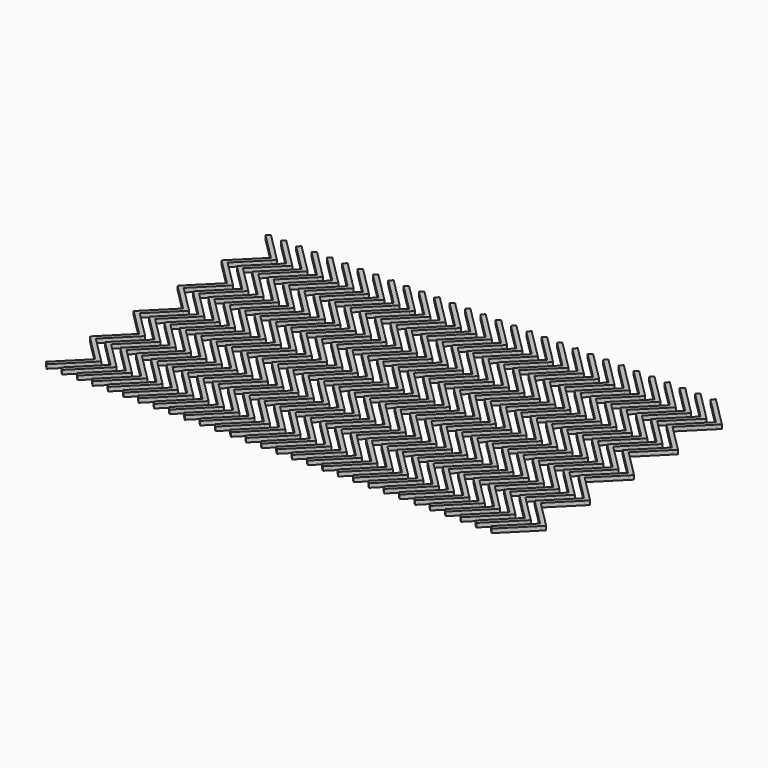
from build123d import *

# Parameters (mm, degrees)
F1_DEPTH = 0.5


with BuildPart() as f1:
    # F0 (on Top) → F1 (new body)
    with BuildSketch(Plane.XY):
        Polygon((-2.3625613103, 20.2585910098), (-1.9869433281, 20.6342089921), (-5.3674577534, 24.0147234175), (-5.7430757357, 23.6391054352), align=None)
        Polygon((-1.9869433281, 13.0829730276), (-2.3625613103, 13.4585910098), (-5.7430757357, 10.0780765845), (-5.7235901611, 10.0585910098), (-5.3674577534, 10.4147234175), (-5.0113253458, 10.0585910098), align=None)
        Polygon((-1.9869433281, 0.2342089921), (-5.0113253458, 3.2585910098), (-5.3674577534, 2.9024586022), (-5.7235901611, 3.2585910098), (-5.7430757357, 3.2391054352), (-2.3625613103, -0.1414089902), align=None)
        Polygon((-1.9869433281, 13.8342089921), (-5.0113253458, 16.8585910098), (-5.3674577534, 16.5024586022), (-5.7235901611, 16.8585910098), (-5.7430757357, 16.8391054352), (-2.3625613103, 13.4585910098), align=None)
        Polygon((-1.9869433281, -6.5657910079), (-5.0113253458, -3.5414089902), (-5.3674577534, -3.8975413978), (-5.7235901611, -3.5414089902), (-5.7430757357, -3.5608945648), (-2.3625613103, -6.9414089902), align=None)
        Polygon((-5.3674577534, 9.7024586022), (-5.0113253458, 10.0585910098), (-5.3674577534, 10.4147234175), (-5.7235901611, 10.0585910098), align=None)
        Polygon((-1.6113253458, -6.9414089902), (-1.9869433281, -6.5657910079), (-2.3625613103, -6.9414089902), (-1.9869433281, -7.3170269724), align=None)
        Polygon((-1.9869433281, -7.3170269724), (-2.3625613103, -6.9414089902), (-5.7430757357, -10.3219234155), (-5.3674577534, -10.6975413978), align=None)
        Polygon((-1.9869433281, -0.5170269724), (-2.3625613103, -0.1414089902), (-5.7430757357, -3.5219234155), (-5.7235901611, -3.5414089902), (-5.3674577534, -3.1852765825), (-5.0113253458, -3.5414089902), align=None)
        Polygon((-5.0113253458, 16.8585910098), (-1.9869433281, 19.8829730276), (-2.3625613103, 20.2585910098), (-5.7430757357, 16.8780765845), (-5.7235901611, 16.8585910098), (-5.3674577534, 17.2147234175), align=None)
        Polygon((-1.9869433281, 6.2829730276), (-2.3625613103, 6.6585910098), (-5.7430757357, 3.2780765845), (-5.7235901611, 3.2585910098), (-5.3674577534, 3.6147234175), (-5.0113253458, 3.2585910098), align=None)
        Polygon((-1.9869433281, 7.0342089921), (-5.0113253458, 10.0585910098), (-5.3674577534, 9.7024586022), (-5.7235901611, 10.0585910098), (-5.7430757357, 10.0391054352), (-2.3625613103, 6.6585910098), align=None)
        Polygon((-5.3674577534, -3.8975413978), (-5.0113253458, -3.5414089902), (-5.3674577534, -3.1852765825), (-5.7235901611, -3.5414089902), align=None)
        Polygon((-5.3674577534, 2.9024586022), (-5.0113253458, 3.2585910098), (-5.3674577534, 3.6147234175), (-5.7235901611, 3.2585910098), align=None)
        Polygon((-1.6113253458, 6.6585910098), (-1.9869433281, 7.0342089921), (-2.3625613103, 6.6585910098), (-1.9869433281, 6.2829730276), align=None)
        Polygon((-5.3674577534, 16.5024586022), (-5.0113253458, 16.8585910098), (-5.3674577534, 17.2147234175), (-5.7235901611, 16.8585910098), align=None)
        Polygon((-1.6113253458, 13.4585910098), (-1.9869433281, 13.8342089921), (-2.3625613103, 13.4585910098), (-1.9869433281, 13.0829730276), align=None)
        Polygon((-1.6113253458, -0.1414089902), (-1.9869433281, 0.2342089921), (-2.3625613103, -0.1414089902), (-1.9869433281, -0.5170269724), align=None)
        Polygon((-1.9869433281, 19.8829730276), (-1.6113253458, 20.2585910098), (-1.9869433281, 20.6342089921), (-2.3625613103, 20.2585910098), align=None)
    extrude(amount=F1_DEPTH)


with BuildPart() as f1b:
    # F0 (on Top) → F1, piece 2 (new body)
    with BuildSketch(Plane.XY):
        Polygon((-4.2625613103, 20.2585910098), (-3.8869433281, 20.6342089921), (-7.2674577534, 24.0147234175), (-7.6430757357, 23.6391054352), align=None)
        Polygon((-3.8869433281, 13.0829730276), (-4.2625613103, 13.4585910098), (-7.6430757357, 10.0780765845), (-7.6235901611, 10.0585910098), (-7.2674577534, 10.4147234175), (-6.9113253458, 10.0585910098), align=None)
        Polygon((-3.8869433281, 0.2342089921), (-6.9113253458, 3.2585910098), (-7.2674577534, 2.9024586022), (-7.6235901611, 3.2585910098), (-7.6430757357, 3.2391054352), (-4.2625613103, -0.1414089902), align=None)
        Polygon((-3.8869433281, -6.5657910079), (-6.9113253458, -3.5414089902), (-7.2674577534, -3.8975413978), (-7.6235901611, -3.5414089902), (-7.6430757357, -3.5608945648), (-4.2625613103, -6.9414089902), align=None)
        Polygon((-3.8869433281, -0.5170269724), (-4.2625613103, -0.1414089902), (-7.6430757357, -3.5219234155), (-7.6235901611, -3.5414089902), (-7.2674577534, -3.1852765825), (-6.9113253458, -3.5414089902), align=None)
        Polygon((-3.8869433281, 13.8342089921), (-6.9113253458, 16.8585910098), (-7.2674577534, 16.5024586022), (-7.6235901611, 16.8585910098), (-7.6430757357, 16.8391054352), (-4.2625613103, 13.4585910098), align=None)
        Polygon((-3.8869433281, 7.0342089921), (-6.9113253458, 10.0585910098), (-7.2674577534, 9.7024586022), (-7.6235901611, 10.0585910098), (-7.6430757357, 10.0391054352), (-4.2625613103, 6.6585910098), align=None)
        Polygon((-6.9113253458, 16.8585910098), (-3.8869433281, 19.8829730276), (-4.2625613103, 20.2585910098), (-7.6430757357, 16.8780765845), (-7.6235901611, 16.8585910098), (-7.2674577534, 17.2147234175), align=None)
        Polygon((-3.8869433281, 6.2829730276), (-4.2625613103, 6.6585910098), (-7.6430757357, 3.2780765845), (-7.6235901611, 3.2585910098), (-7.2674577534, 3.6147234175), (-6.9113253458, 3.2585910098), align=None)
        Polygon((-7.2674577534, 16.5024586022), (-6.9113253458, 16.8585910098), (-7.2674577534, 17.2147234175), (-7.6235901611, 16.8585910098), align=None)
        Polygon((-3.5113253458, -6.9414089902), (-3.8869433281, -6.5657910079), (-4.2625613103, -6.9414089902), (-3.8869433281, -7.3170269724), align=None)
        Polygon((-3.8869433281, -7.3170269724), (-4.2625613103, -6.9414089902), (-7.6430757357, -10.3219234155), (-7.2674577534, -10.6975413978), align=None)
        Polygon((-7.2674577534, 9.7024586022), (-6.9113253458, 10.0585910098), (-7.2674577534, 10.4147234175), (-7.6235901611, 10.0585910098), align=None)
        Polygon((-7.2674577534, -3.8975413978), (-6.9113253458, -3.5414089902), (-7.2674577534, -3.1852765825), (-7.6235901611, -3.5414089902), align=None)
        Polygon((-3.5113253458, 6.6585910098), (-3.8869433281, 7.0342089921), (-4.2625613103, 6.6585910098), (-3.8869433281, 6.2829730276), align=None)
        Polygon((-7.2674577534, 2.9024586022), (-6.9113253458, 3.2585910098), (-7.2674577534, 3.6147234175), (-7.6235901611, 3.2585910098), align=None)
        Polygon((-3.8869433281, 19.8829730276), (-3.5113253458, 20.2585910098), (-3.8869433281, 20.6342089921), (-4.2625613103, 20.2585910098), align=None)
        Polygon((-3.5113253458, 13.4585910098), (-3.8869433281, 13.8342089921), (-4.2625613103, 13.4585910098), (-3.8869433281, 13.0829730276), align=None)
        Polygon((-3.5113253458, -0.1414089902), (-3.8869433281, 0.2342089921), (-4.2625613103, -0.1414089902), (-3.8869433281, -0.5170269724), align=None)
    extrude(amount=F1_DEPTH)


with BuildPart() as f1c:
    # F0 (on Top) → F1, piece 3 (new body)
    with BuildSketch(Plane.XY):
        Polygon((-8.0625613103, 20.2585910098), (-7.6869433281, 20.6342089921), (-11.0674577534, 24.0147234175), (-11.4430757357, 23.6391054352), align=None)
        Polygon((-7.6869433281, 0.2342089921), (-10.7113253458, 3.2585910098), (-11.0674577534, 2.9024586022), (-11.4235901611, 3.2585910098), (-11.4430757357, 3.2391054352), (-8.0625613103, -0.1414089902), align=None)
        Polygon((-7.6869433281, 13.0829730276), (-8.0625613103, 13.4585910098), (-11.4430757357, 10.0780765845), (-11.4235901611, 10.0585910098), (-11.0674577534, 10.4147234175), (-10.7113253458, 10.0585910098), align=None)
        Polygon((-7.6869433281, 13.8342089921), (-10.7113253458, 16.8585910098), (-11.0674577534, 16.5024586022), (-11.4235901611, 16.8585910098), (-11.4430757357, 16.8391054352), (-8.0625613103, 13.4585910098), align=None)
        Polygon((-7.6869433281, 6.2829730276), (-8.0625613103, 6.6585910098), (-11.4430757357, 3.2780765845), (-11.4235901611, 3.2585910098), (-11.0674577534, 3.6147234175), (-10.7113253458, 3.2585910098), align=None)
        Polygon((-7.6869433281, -7.3170269724), (-8.0625613103, -6.9414089902), (-11.4430757357, -10.3219234155), (-11.0674577534, -10.6975413978), align=None)
        Polygon((-7.6869433281, 7.0342089921), (-10.7113253458, 10.0585910098), (-11.0674577534, 9.7024586022), (-11.4235901611, 10.0585910098), (-11.4430757357, 10.0391054352), (-8.0625613103, 6.6585910098), align=None)
        Polygon((-7.3113253458, 6.6585910098), (-7.6869433281, 7.0342089921), (-8.0625613103, 6.6585910098), (-7.6869433281, 6.2829730276), align=None)
        Polygon((-10.7113253458, 16.8585910098), (-7.6869433281, 19.8829730276), (-8.0625613103, 20.2585910098), (-11.4430757357, 16.8780765845), (-11.4235901611, 16.8585910098), (-11.0674577534, 17.2147234175), align=None)
        Polygon((-11.0674577534, 16.5024586022), (-10.7113253458, 16.8585910098), (-11.0674577534, 17.2147234175), (-11.4235901611, 16.8585910098), align=None)
        Polygon((-7.6869433281, -0.5170269724), (-8.0625613103, -0.1414089902), (-11.4430757357, -3.5219234155), (-11.4235901611, -3.5414089902), (-11.0674577534, -3.1852765825), (-10.7113253458, -3.5414089902), align=None)
        Polygon((-11.0674577534, 9.7024586022), (-10.7113253458, 10.0585910098), (-11.0674577534, 10.4147234175), (-11.4235901611, 10.0585910098), align=None)
        Polygon((-7.6869433281, -6.5657910079), (-10.7113253458, -3.5414089902), (-11.0674577534, -3.8975413978), (-11.4235901611, -3.5414089902), (-11.4430757357, -3.5608945648), (-8.0625613103, -6.9414089902), align=None)
        Polygon((-11.0674577534, 2.9024586022), (-10.7113253458, 3.2585910098), (-11.0674577534, 3.6147234175), (-11.4235901611, 3.2585910098), align=None)
        Polygon((-7.3113253458, -0.1414089902), (-7.6869433281, 0.2342089921), (-8.0625613103, -0.1414089902), (-7.6869433281, -0.5170269724), align=None)
        Polygon((-7.3113253458, -6.9414089902), (-7.6869433281, -6.5657910079), (-8.0625613103, -6.9414089902), (-7.6869433281, -7.3170269724), align=None)
        Polygon((-11.0674577534, -3.8975413978), (-10.7113253458, -3.5414089902), (-11.0674577534, -3.1852765825), (-11.4235901611, -3.5414089902), align=None)
        Polygon((-7.3113253458, 13.4585910098), (-7.6869433281, 13.8342089921), (-8.0625613103, 13.4585910098), (-7.6869433281, 13.0829730276), align=None)
        Polygon((-7.6869433281, 19.8829730276), (-7.3113253458, 20.2585910098), (-7.6869433281, 20.6342089921), (-8.0625613103, 20.2585910098), align=None)
    extrude(amount=F1_DEPTH)


with BuildPart() as f1d:
    # F0 (on Top) → F1, piece 4 (new body)
    with BuildSketch(Plane.XY):
        Polygon((-9.9625613103, 20.2585910098), (-9.5869433281, 20.6342089921), (-12.9674577534, 24.0147234175), (-13.3430757357, 23.6391054352), align=None)
        Polygon((-9.5869433281, 13.0829730276), (-9.9625613103, 13.4585910098), (-13.3430757357, 10.0780765845), (-13.3235901611, 10.0585910098), (-12.9674577534, 10.4147234175), (-12.6113253458, 10.0585910098), align=None)
        Polygon((-9.5869433281, 0.2342089921), (-12.6113253458, 3.2585910098), (-12.9674577534, 2.9024586022), (-13.3235901611, 3.2585910098), (-13.3430757357, 3.2391054352), (-9.9625613103, -0.1414089902), align=None)
        Polygon((-9.5869433281, -7.3170269724), (-9.9625613103, -6.9414089902), (-13.3430757357, -10.3219234155), (-12.9674577534, -10.6975413978), align=None)
        Polygon((-9.5869433281, -0.5170269724), (-9.9625613103, -0.1414089902), (-13.3430757357, -3.5219234155), (-13.3235901611, -3.5414089902), (-12.9674577534, -3.1852765825), (-12.6113253458, -3.5414089902), align=None)
        Polygon((-9.5869433281, 6.2829730276), (-9.9625613103, 6.6585910098), (-13.3430757357, 3.2780765845), (-13.3235901611, 3.2585910098), (-12.9674577534, 3.6147234175), (-12.6113253458, 3.2585910098), align=None)
        Polygon((-9.5869433281, 7.0342089921), (-12.6113253458, 10.0585910098), (-12.9674577534, 9.7024586022), (-13.3235901611, 10.0585910098), (-13.3430757357, 10.0391054352), (-9.9625613103, 6.6585910098), align=None)
        Polygon((-9.5869433281, 13.8342089921), (-12.6113253458, 16.8585910098), (-12.9674577534, 16.5024586022), (-13.3235901611, 16.8585910098), (-13.3430757357, 16.8391054352), (-9.9625613103, 13.4585910098), align=None)
        Polygon((-9.5869433281, -6.5657910079), (-12.6113253458, -3.5414089902), (-12.9674577534, -3.8975413978), (-13.3235901611, -3.5414089902), (-13.3430757357, -3.5608945648), (-9.9625613103, -6.9414089902), align=None)
        Polygon((-12.6113253458, 16.8585910098), (-9.5869433281, 19.8829730276), (-9.9625613103, 20.2585910098), (-13.3430757357, 16.8780765845), (-13.3235901611, 16.8585910098), (-12.9674577534, 17.2147234175), align=None)
        Polygon((-9.2113253458, -6.9414089902), (-9.5869433281, -6.5657910079), (-9.9625613103, -6.9414089902), (-9.5869433281, -7.3170269724), align=None)
        Polygon((-12.9674577534, 2.9024586022), (-12.6113253458, 3.2585910098), (-12.9674577534, 3.6147234175), (-13.3235901611, 3.2585910098), align=None)
        Polygon((-9.2113253458, 6.6585910098), (-9.5869433281, 7.0342089921), (-9.9625613103, 6.6585910098), (-9.5869433281, 6.2829730276), align=None)
        Polygon((-12.9674577534, 9.7024586022), (-12.6113253458, 10.0585910098), (-12.9674577534, 10.4147234175), (-13.3235901611, 10.0585910098), align=None)
        Polygon((-12.9674577534, -3.8975413978), (-12.6113253458, -3.5414089902), (-12.9674577534, -3.1852765825), (-13.3235901611, -3.5414089902), align=None)
        Polygon((-12.9674577534, 16.5024586022), (-12.6113253458, 16.8585910098), (-12.9674577534, 17.2147234175), (-13.3235901611, 16.8585910098), align=None)
        Polygon((-9.2113253458, 13.4585910098), (-9.5869433281, 13.8342089921), (-9.9625613103, 13.4585910098), (-9.5869433281, 13.0829730276), align=None)
        Polygon((-9.5869433281, 19.8829730276), (-9.2113253458, 20.2585910098), (-9.5869433281, 20.6342089921), (-9.9625613103, 20.2585910098), align=None)
        Polygon((-9.2113253458, -0.1414089902), (-9.5869433281, 0.2342089921), (-9.9625613103, -0.1414089902), (-9.5869433281, -0.5170269724), align=None)
    extrude(amount=F1_DEPTH)


with BuildPart() as f1e:
    # F0 (on Top) → F1, piece 5 (new body)
    with BuildSketch(Plane.XY):
        Polygon((-17.5625613103, 20.2585910098), (-17.1869433281, 20.6342089921), (-20.5674577534, 24.0147234175), (-20.9430757357, 23.6391054352), align=None)
        Polygon((-17.1869433281, 13.0829730276), (-17.5625613103, 13.4585910098), (-20.9430757357, 10.0780765845), (-20.9235901611, 10.0585910098), (-20.5674577534, 10.4147234175), (-20.2113253458, 10.0585910098), align=None)
        Polygon((-17.1869433281, 0.2342089921), (-20.2113253458, 3.2585910098), (-20.5674577534, 2.9024586022), (-20.9235901611, 3.2585910098), (-20.9430757357, 3.2391054352), (-17.5625613103, -0.1414089902), align=None)
        Polygon((-17.1869433281, -0.5170269724), (-17.5625613103, -0.1414089902), (-20.9430757357, -3.5219234155), (-20.9235901611, -3.5414089902), (-20.5674577534, -3.1852765825), (-20.2113253458, -3.5414089902), align=None)
        Polygon((-17.1869433281, 7.0342089921), (-20.2113253458, 10.0585910098), (-20.5674577534, 9.7024586022), (-20.9235901611, 10.0585910098), (-20.9430757357, 10.0391054352), (-17.5625613103, 6.6585910098), align=None)
        Polygon((-17.1869433281, -7.3170269724), (-17.5625613103, -6.9414089902), (-20.9430757357, -10.3219234155), (-20.5674577534, -10.6975413978), align=None)
        Polygon((-16.8113253458, -0.1414089902), (-17.1869433281, 0.2342089921), (-17.5625613103, -0.1414089902), (-17.1869433281, -0.5170269724), align=None)
        Polygon((-17.1869433281, 6.2829730276), (-17.5625613103, 6.6585910098), (-20.9430757357, 3.2780765845), (-20.9235901611, 3.2585910098), (-20.5674577534, 3.6147234175), (-20.2113253458, 3.2585910098), align=None)
        Polygon((-17.1869433281, -6.5657910079), (-20.2113253458, -3.5414089902), (-20.5674577534, -3.8975413978), (-20.9235901611, -3.5414089902), (-20.9430757357, -3.5608945648), (-17.5625613103, -6.9414089902), align=None)
        Polygon((-20.5674577534, 9.7024586022), (-20.2113253458, 10.0585910098), (-20.5674577534, 10.4147234175), (-20.9235901611, 10.0585910098), align=None)
        Polygon((-20.2113253458, 16.8585910098), (-17.1869433281, 19.8829730276), (-17.5625613103, 20.2585910098), (-20.9430757357, 16.8780765845), (-20.9235901611, 16.8585910098), (-20.5674577534, 17.2147234175), align=None)
        Polygon((-17.1869433281, 13.8342089921), (-20.2113253458, 16.8585910098), (-20.5674577534, 16.5024586022), (-20.9235901611, 16.8585910098), (-20.9430757357, 16.8391054352), (-17.5625613103, 13.4585910098), align=None)
        Polygon((-16.8113253458, -6.9414089902), (-17.1869433281, -6.5657910079), (-17.5625613103, -6.9414089902), (-17.1869433281, -7.3170269724), align=None)
        Polygon((-16.8113253458, 13.4585910098), (-17.1869433281, 13.8342089921), (-17.5625613103, 13.4585910098), (-17.1869433281, 13.0829730276), align=None)
        Polygon((-20.5674577534, 2.9024586022), (-20.2113253458, 3.2585910098), (-20.5674577534, 3.6147234175), (-20.9235901611, 3.2585910098), align=None)
        Polygon((-16.8113253458, 6.6585910098), (-17.1869433281, 7.0342089921), (-17.5625613103, 6.6585910098), (-17.1869433281, 6.2829730276), align=None)
        Polygon((-20.5674577534, -3.8975413978), (-20.2113253458, -3.5414089902), (-20.5674577534, -3.1852765825), (-20.9235901611, -3.5414089902), align=None)
        Polygon((-20.5674577534, 16.5024586022), (-20.2113253458, 16.8585910098), (-20.5674577534, 17.2147234175), (-20.9235901611, 16.8585910098), align=None)
        Polygon((-17.1869433281, 19.8829730276), (-16.8113253458, 20.2585910098), (-17.1869433281, 20.6342089921), (-17.5625613103, 20.2585910098), align=None)
    extrude(amount=F1_DEPTH)


with BuildPart() as f1f:
    # F0 (on Top) → F1, piece 6 (new body)
    with BuildSketch(Plane.XY):
        Polygon((-19.4625613103, 20.2585910098), (-19.0869433281, 20.6342089921), (-22.4674577534, 24.0147234175), (-22.8430757357, 23.6391054352), align=None)
        Polygon((-19.0869433281, 13.0829730276), (-19.4625613103, 13.4585910098), (-22.8430757357, 10.0780765845), (-22.8235901611, 10.0585910098), (-22.4674577534, 10.4147234175), (-22.1113253458, 10.0585910098), align=None)
        Polygon((-19.0869433281, 0.2342089921), (-22.1113253458, 3.2585910098), (-22.4674577534, 2.9024586022), (-22.8235901611, 3.2585910098), (-22.8430757357, 3.2391054352), (-19.4625613103, -0.1414089902), align=None)
        Polygon((-19.0869433281, 6.2829730276), (-19.4625613103, 6.6585910098), (-22.8430757357, 3.2780765845), (-22.8235901611, 3.2585910098), (-22.4674577534, 3.6147234175), (-22.1113253458, 3.2585910098), align=None)
        Polygon((-19.0869433281, 7.0342089921), (-22.1113253458, 10.0585910098), (-22.4674577534, 9.7024586022), (-22.8235901611, 10.0585910098), (-22.8430757357, 10.0391054352), (-19.4625613103, 6.6585910098), align=None)
        Polygon((-19.0869433281, -6.5657910079), (-22.1113253458, -3.5414089902), (-22.4674577534, -3.8975413978), (-22.8235901611, -3.5414089902), (-22.8430757357, -3.5608945648), (-19.4625613103, -6.9414089902), align=None)
        Polygon((-19.0869433281, 13.8342089921), (-22.1113253458, 16.8585910098), (-22.4674577534, 16.5024586022), (-22.8235901611, 16.8585910098), (-22.8430757357, 16.8391054352), (-19.4625613103, 13.4585910098), align=None)
        Polygon((-19.0869433281, -0.5170269724), (-19.4625613103, -0.1414089902), (-22.8430757357, -3.5219234155), (-22.8235901611, -3.5414089902), (-22.4674577534, -3.1852765825), (-22.1113253458, -3.5414089902), align=None)
        Polygon((-19.0869433281, -7.3170269724), (-19.4625613103, -6.9414089902), (-22.8430757357, -10.3219234155), (-22.4674577534, -10.6975413978), align=None)
        Polygon((-22.4674577534, 9.7024586022), (-22.1113253458, 10.0585910098), (-22.4674577534, 10.4147234175), (-22.8235901611, 10.0585910098), align=None)
        Polygon((-18.7113253458, 6.6585910098), (-19.0869433281, 7.0342089921), (-19.4625613103, 6.6585910098), (-19.0869433281, 6.2829730276), align=None)
        Polygon((-22.1113253458, 16.8585910098), (-19.0869433281, 19.8829730276), (-19.4625613103, 20.2585910098), (-22.8430757357, 16.8780765845), (-22.8235901611, 16.8585910098), (-22.4674577534, 17.2147234175), align=None)
        Polygon((-22.4674577534, 16.5024586022), (-22.1113253458, 16.8585910098), (-22.4674577534, 17.2147234175), (-22.8235901611, 16.8585910098), align=None)
        Polygon((-18.7113253458, -6.9414089902), (-19.0869433281, -6.5657910079), (-19.4625613103, -6.9414089902), (-19.0869433281, -7.3170269724), align=None)
        Polygon((-22.4674577534, -3.8975413978), (-22.1113253458, -3.5414089902), (-22.4674577534, -3.1852765825), (-22.8235901611, -3.5414089902), align=None)
        Polygon((-19.0869433281, 19.8829730276), (-18.7113253458, 20.2585910098), (-19.0869433281, 20.6342089921), (-19.4625613103, 20.2585910098), align=None)
        Polygon((-22.4674577534, 2.9024586022), (-22.1113253458, 3.2585910098), (-22.4674577534, 3.6147234175), (-22.8235901611, 3.2585910098), align=None)
        Polygon((-18.7113253458, -0.1414089902), (-19.0869433281, 0.2342089921), (-19.4625613103, -0.1414089902), (-19.0869433281, -0.5170269724), align=None)
        Polygon((-18.7113253458, 13.4585910098), (-19.0869433281, 13.8342089921), (-19.4625613103, 13.4585910098), (-19.0869433281, 13.0829730276), align=None)
    extrude(amount=F1_DEPTH)


with BuildPart() as f1g:
    # F0 (on Top) → F1, piece 7 (new body)
    with BuildSketch(Plane.XY):
        Polygon((-21.3625613103, 20.2585910098), (-20.9869433281, 20.6342089921), (-24.3674577534, 24.0147234175), (-24.7430757357, 23.6391054352), align=None)
        Polygon((-20.9869433281, 0.2342089921), (-24.0113253458, 3.2585910098), (-24.3674577534, 2.9024586022), (-24.7235901611, 3.2585910098), (-24.7430757357, 3.2391054352), (-21.3625613103, -0.1414089902), align=None)
        Polygon((-20.9869433281, 13.0829730276), (-21.3625613103, 13.4585910098), (-24.7430757357, 10.0780765845), (-24.7235901611, 10.0585910098), (-24.3674577534, 10.4147234175), (-24.0113253458, 10.0585910098), align=None)
        Polygon((-20.9869433281, 13.8342089921), (-24.0113253458, 16.8585910098), (-24.3674577534, 16.5024586022), (-24.7235901611, 16.8585910098), (-24.7430757357, 16.8391054352), (-21.3625613103, 13.4585910098), align=None)
        Polygon((-20.9869433281, -7.3170269724), (-21.3625613103, -6.9414089902), (-24.7430757357, -10.3219234155), (-24.3674577534, -10.6975413978), align=None)
        Polygon((-20.9869433281, -0.5170269724), (-21.3625613103, -0.1414089902), (-24.7430757357, -3.5219234155), (-24.7235901611, -3.5414089902), (-24.3674577534, -3.1852765825), (-24.0113253458, -3.5414089902), align=None)
        Polygon((-20.9869433281, -6.5657910079), (-24.0113253458, -3.5414089902), (-24.3674577534, -3.8975413978), (-24.7235901611, -3.5414089902), (-24.7430757357, -3.5608945648), (-21.3625613103, -6.9414089902), align=None)
        Polygon((-20.9869433281, 6.2829730276), (-21.3625613103, 6.6585910098), (-24.7430757357, 3.2780765845), (-24.7235901611, 3.2585910098), (-24.3674577534, 3.6147234175), (-24.0113253458, 3.2585910098), align=None)
        Polygon((-24.0113253458, 16.8585910098), (-20.9869433281, 19.8829730276), (-21.3625613103, 20.2585910098), (-24.7430757357, 16.8780765845), (-24.7235901611, 16.8585910098), (-24.3674577534, 17.2147234175), align=None)
        Polygon((-20.9869433281, 7.0342089921), (-24.0113253458, 10.0585910098), (-24.3674577534, 9.7024586022), (-24.7235901611, 10.0585910098), (-24.7430757357, 10.0391054352), (-21.3625613103, 6.6585910098), align=None)
        Polygon((-20.6113253458, -6.9414089902), (-20.9869433281, -6.5657910079), (-21.3625613103, -6.9414089902), (-20.9869433281, -7.3170269724), align=None)
        Polygon((-20.9869433281, 19.8829730276), (-20.6113253458, 20.2585910098), (-20.9869433281, 20.6342089921), (-21.3625613103, 20.2585910098), align=None)
        Polygon((-24.3674577534, 16.5024586022), (-24.0113253458, 16.8585910098), (-24.3674577534, 17.2147234175), (-24.7235901611, 16.8585910098), align=None)
        Polygon((-20.6113253458, 6.6585910098), (-20.9869433281, 7.0342089921), (-21.3625613103, 6.6585910098), (-20.9869433281, 6.2829730276), align=None)
        Polygon((-24.3674577534, 9.7024586022), (-24.0113253458, 10.0585910098), (-24.3674577534, 10.4147234175), (-24.7235901611, 10.0585910098), align=None)
        Polygon((-20.6113253458, 13.4585910098), (-20.9869433281, 13.8342089921), (-21.3625613103, 13.4585910098), (-20.9869433281, 13.0829730276), align=None)
        Polygon((-24.3674577534, 2.9024586022), (-24.0113253458, 3.2585910098), (-24.3674577534, 3.6147234175), (-24.7235901611, 3.2585910098), align=None)
        Polygon((-20.6113253458, -0.1414089902), (-20.9869433281, 0.2342089921), (-21.3625613103, -0.1414089902), (-20.9869433281, -0.5170269724), align=None)
        Polygon((-24.3674577534, -3.8975413978), (-24.0113253458, -3.5414089902), (-24.3674577534, -3.1852765825), (-24.7235901611, -3.5414089902), align=None)
    extrude(amount=F1_DEPTH)


with BuildPart() as f1h:
    # F0 (on Top) → F1, piece 8 (new body)
    with BuildSketch(Plane.XY):
        Polygon((-23.2625613103, 20.2585910098), (-22.8869433281, 20.6342089921), (-26.2674577534, 24.0147234175), (-26.6430757357, 23.6391054352), align=None)
        Polygon((-25.9113253458, 16.8585910098), (-22.8869433281, 19.8829730276), (-23.2625613103, 20.2585910098), (-26.6430757357, 16.8780765845), (-26.6235901611, 16.8585910098), (-26.2674577534, 17.2147234175), align=None)
        Polygon((-22.8869433281, 6.2829730276), (-23.2625613103, 6.6585910098), (-26.6430757357, 3.2780765845), (-26.6235901611, 3.2585910098), (-26.2674577534, 3.6147234175), (-25.9113253458, 3.2585910098), align=None)
        Polygon((-22.8869433281, 13.8342089921), (-25.9113253458, 16.8585910098), (-26.2674577534, 16.5024586022), (-26.6235901611, 16.8585910098), (-26.6430757357, 16.8391054352), (-23.2625613103, 13.4585910098), align=None)
        Polygon((-22.8869433281, 0.2342089921), (-25.9113253458, 3.2585910098), (-26.2674577534, 2.9024586022), (-26.6235901611, 3.2585910098), (-26.6430757357, 3.2391054352), (-23.2625613103, -0.1414089902), align=None)
        Polygon((-22.8869433281, 13.0829730276), (-23.2625613103, 13.4585910098), (-26.6430757357, 10.0780765845), (-26.6235901611, 10.0585910098), (-26.2674577534, 10.4147234175), (-25.9113253458, 10.0585910098), align=None)
        Polygon((-22.8869433281, -0.5170269724), (-23.2625613103, -0.1414089902), (-26.6430757357, -3.5219234155), (-26.6235901611, -3.5414089902), (-26.2674577534, -3.1852765825), (-25.9113253458, -3.5414089902), align=None)
        Polygon((-22.8869433281, -6.5657910079), (-25.9113253458, -3.5414089902), (-26.2674577534, -3.8975413978), (-26.6235901611, -3.5414089902), (-26.6430757357, -3.5608945648), (-23.2625613103, -6.9414089902), align=None)
        Polygon((-22.8869433281, 7.0342089921), (-25.9113253458, 10.0585910098), (-26.2674577534, 9.7024586022), (-26.6235901611, 10.0585910098), (-26.6430757357, 10.0391054352), (-23.2625613103, 6.6585910098), align=None)
        Polygon((-22.8869433281, -7.3170269724), (-23.2625613103, -6.9414089902), (-26.6430757357, -10.3219234155), (-26.2674577534, -10.6975413978), align=None)
        Polygon((-26.2674577534, 16.5024586022), (-25.9113253458, 16.8585910098), (-26.2674577534, 17.2147234175), (-26.6235901611, 16.8585910098), align=None)
        Polygon((-22.5113253458, 13.4585910098), (-22.8869433281, 13.8342089921), (-23.2625613103, 13.4585910098), (-22.8869433281, 13.0829730276), align=None)
        Polygon((-22.5113253458, -0.1414089902), (-22.8869433281, 0.2342089921), (-23.2625613103, -0.1414089902), (-22.8869433281, -0.5170269724), align=None)
        Polygon((-22.5113253458, 6.6585910098), (-22.8869433281, 7.0342089921), (-23.2625613103, 6.6585910098), (-22.8869433281, 6.2829730276), align=None)
        Polygon((-26.2674577534, 2.9024586022), (-25.9113253458, 3.2585910098), (-26.2674577534, 3.6147234175), (-26.6235901611, 3.2585910098), align=None)
        Polygon((-26.2674577534, -3.8975413978), (-25.9113253458, -3.5414089902), (-26.2674577534, -3.1852765825), (-26.6235901611, -3.5414089902), align=None)
        Polygon((-22.5113253458, -6.9414089902), (-22.8869433281, -6.5657910079), (-23.2625613103, -6.9414089902), (-22.8869433281, -7.3170269724), align=None)
        Polygon((-22.8869433281, 19.8829730276), (-22.5113253458, 20.2585910098), (-22.8869433281, 20.6342089921), (-23.2625613103, 20.2585910098), align=None)
        Polygon((-26.2674577534, 9.7024586022), (-25.9113253458, 10.0585910098), (-26.2674577534, 10.4147234175), (-26.6235901611, 10.0585910098), align=None)
    extrude(amount=F1_DEPTH)


with BuildPart() as f1i:
    # F0 (on Top) → F1, piece 9 (new body)
    with BuildSketch(Plane.XY):
        Polygon((5.2374386897, 20.2585910098), (5.6130566719, 20.6342089921), (2.2325422466, 24.0147234175), (1.8569242643, 23.6391054352), align=None)
        Polygon((5.6130566719, 0.2342089921), (2.5886746542, 3.2585910098), (2.2325422466, 2.9024586022), (1.8764098389, 3.2585910098), (1.8569242643, 3.2391054352), (5.2374386897, -0.1414089902), align=None)
        Polygon((5.6130566719, 13.0829730276), (5.2374386897, 13.4585910098), (1.8569242643, 10.0780765845), (1.8764098389, 10.0585910098), (2.2325422466, 10.4147234175), (2.5886746542, 10.0585910098), align=None)
        Polygon((5.6130566719, 7.0342089921), (2.5886746542, 10.0585910098), (2.2325422466, 9.7024586022), (1.8764098389, 10.0585910098), (1.8569242643, 10.0391054352), (5.2374386897, 6.6585910098), align=None)
        Polygon((5.6130566719, 6.2829730276), (5.2374386897, 6.6585910098), (1.8569242643, 3.2780765845), (1.8764098389, 3.2585910098), (2.2325422466, 3.6147234175), (2.5886746542, 3.2585910098), align=None)
        Polygon((5.6130566719, -7.3170269724), (5.2374386897, -6.9414089902), (1.8569242643, -10.3219234155), (2.2325422466, -10.6975413978), align=None)
        Polygon((5.6130566719, -0.5170269724), (5.2374386897, -0.1414089902), (1.8569242643, -3.5219234155), (1.8764098389, -3.5414089902), (2.2325422466, -3.1852765825), (2.5886746542, -3.5414089902), align=None)
        Polygon((5.6130566719, -6.5657910079), (2.5886746542, -3.5414089902), (2.2325422466, -3.8975413978), (1.8764098389, -3.5414089902), (1.8569242643, -3.5608945648), (5.2374386897, -6.9414089902), align=None)
        Polygon((2.5886746542, 16.8585910098), (5.6130566719, 19.8829730276), (5.2374386897, 20.2585910098), (1.8569242643, 16.8780765845), (1.8764098389, 16.8585910098), (2.2325422466, 17.2147234175), align=None)
        Polygon((5.6130566719, 13.8342089921), (2.5886746542, 16.8585910098), (2.2325422466, 16.5024586022), (1.8764098389, 16.8585910098), (1.8569242643, 16.8391054352), (5.2374386897, 13.4585910098), align=None)
        Polygon((5.9886746542, -6.9414089902), (5.6130566719, -6.5657910079), (5.2374386897, -6.9414089902), (5.6130566719, -7.3170269724), align=None)
        Polygon((2.2325422466, 2.9024586022), (2.5886746542, 3.2585910098), (2.2325422466, 3.6147234175), (1.8764098389, 3.2585910098), align=None)
        Polygon((5.9886746542, 6.6585910098), (5.6130566719, 7.0342089921), (5.2374386897, 6.6585910098), (5.6130566719, 6.2829730276), align=None)
        Polygon((2.2325422466, 9.7024586022), (2.5886746542, 10.0585910098), (2.2325422466, 10.4147234175), (1.8764098389, 10.0585910098), align=None)
        Polygon((2.2325422466, -3.8975413978), (2.5886746542, -3.5414089902), (2.2325422466, -3.1852765825), (1.8764098389, -3.5414089902), align=None)
        Polygon((2.2325422466, 16.5024586022), (2.5886746542, 16.8585910098), (2.2325422466, 17.2147234175), (1.8764098389, 16.8585910098), align=None)
        Polygon((5.9886746542, 13.4585910098), (5.6130566719, 13.8342089921), (5.2374386897, 13.4585910098), (5.6130566719, 13.0829730276), align=None)
        Polygon((5.9886746542, -0.1414089902), (5.6130566719, 0.2342089921), (5.2374386897, -0.1414089902), (5.6130566719, -0.5170269724), align=None)
        Polygon((5.6130566719, 19.8829730276), (5.9886746542, 20.2585910098), (5.6130566719, 20.6342089921), (5.2374386897, 20.2585910098), align=None)
    extrude(amount=F1_DEPTH)


with BuildPart() as f1j:
    # F0 (on Top) → F1, piece 10 (new body)
    with BuildSketch(Plane.XY):
        Polygon((32.2130566719, -7.3170269724), (31.8374386897, -6.9414089902), (28.4569242643, -10.3219234155), (28.8325422466, -10.6975413978), align=None)
        Polygon((31.8374386897, 20.2585910098), (32.2130566719, 20.6342089921), (28.8325422466, 24.0147234175), (28.4569242643, 23.6391054352), align=None)
        Polygon((32.2130566719, 6.2829730276), (31.8374386897, 6.6585910098), (28.4569242643, 3.2780765845), (28.4764098389, 3.2585910098), (28.8325422466, 3.6147234175), (29.1886746542, 3.2585910098), align=None)
        Polygon((32.2130566719, 0.2342089921), (29.1886746542, 3.2585910098), (28.8325422466, 2.9024586022), (28.4764098389, 3.2585910098), (28.4569242643, 3.2391054352), (31.8374386897, -0.1414089902), align=None)
        Polygon((29.1886746542, 16.8585910098), (32.2130566719, 19.8829730276), (31.8374386897, 20.2585910098), (28.4569242643, 16.8780765845), (28.4764098389, 16.8585910098), (28.8325422466, 17.2147234175), align=None)
        Polygon((32.2130566719, 13.8342089921), (29.1886746542, 16.8585910098), (28.8325422466, 16.5024586022), (28.4764098389, 16.8585910098), (28.4569242643, 16.8391054352), (31.8374386897, 13.4585910098), align=None)
        Polygon((32.2130566719, 13.0829730276), (31.8374386897, 13.4585910098), (28.4569242643, 10.0780765845), (28.4764098389, 10.0585910098), (28.8325422466, 10.4147234175), (29.1886746542, 10.0585910098), align=None)
        Polygon((32.2130566719, -0.5170269724), (31.8374386897, -0.1414089902), (28.4569242643, -3.5219234155), (28.4764098389, -3.5414089902), (28.8325422466, -3.1852765825), (29.1886746542, -3.5414089902), align=None)
        Polygon((32.2130566719, -6.5657910079), (29.1886746542, -3.5414089902), (28.8325422466, -3.8975413978), (28.4764098389, -3.5414089902), (28.4569242643, -3.5608945648), (31.8374386897, -6.9414089902), align=None)
        Polygon((32.2130566719, 7.0342089921), (29.1886746542, 10.0585910098), (28.8325422466, 9.7024586022), (28.4764098389, 10.0585910098), (28.4569242643, 10.0391054352), (31.8374386897, 6.6585910098), align=None)
        Polygon((32.5886746542, -6.9414089902), (32.2130566719, -6.5657910079), (31.8374386897, -6.9414089902), (32.2130566719, -7.3170269724), align=None)
        Polygon((28.8325422466, 16.5024586022), (29.1886746542, 16.8585910098), (28.8325422466, 17.2147234175), (28.4764098389, 16.8585910098), align=None)
        Polygon((32.5886746542, 6.6585910098), (32.2130566719, 7.0342089921), (31.8374386897, 6.6585910098), (32.2130566719, 6.2829730276), align=None)
        Polygon((32.2130566719, 19.8829730276), (32.5886746542, 20.2585910098), (32.2130566719, 20.6342089921), (31.8374386897, 20.2585910098), align=None)
        Polygon((28.8325422466, 2.9024586022), (29.1886746542, 3.2585910098), (28.8325422466, 3.6147234175), (28.4764098389, 3.2585910098), align=None)
        Polygon((32.5886746542, 13.4585910098), (32.2130566719, 13.8342089921), (31.8374386897, 13.4585910098), (32.2130566719, 13.0829730276), align=None)
        Polygon((32.5886746542, -0.1414089902), (32.2130566719, 0.2342089921), (31.8374386897, -0.1414089902), (32.2130566719, -0.5170269724), align=None)
        Polygon((28.8325422466, -3.8975413978), (29.1886746542, -3.5414089902), (28.8325422466, -3.1852765825), (28.4764098389, -3.5414089902), align=None)
        Polygon((28.8325422466, 9.7024586022), (29.1886746542, 10.0585910098), (28.8325422466, 10.4147234175), (28.4764098389, 10.0585910098), align=None)
    extrude(amount=F1_DEPTH)


with BuildPart() as f1k:
    # F0 (on Top) → F1, piece 11 (new body)
    with BuildSketch(Plane.XY):
        Polygon((7.5130566719, 13.0829730276), (7.1374386897, 13.4585910098), (3.7569242643, 10.0780765845), (3.7764098389, 10.0585910098), (4.1325422466, 10.4147234175), (4.4886746542, 10.0585910098), align=None)
        Polygon((7.1374386897, 20.2585910098), (7.5130566719, 20.6342089921), (4.1325422466, 24.0147234175), (3.7569242643, 23.6391054352), align=None)
        Polygon((4.1325422466, 2.9024586022), (3.7764098389, 3.2585910098), (3.7569242643, 3.2391054352), (7.1374386897, -0.1414089902), (7.5130566719, 0.2342089921), (4.4886746542, 3.2585910098), align=None)
        Polygon((7.5130566719, 13.8342089921), (4.4886746542, 16.8585910098), (4.1325422466, 16.5024586022), (3.7764098389, 16.8585910098), (3.7569242643, 16.8391054352), (7.1374386897, 13.4585910098), align=None)
        Polygon((7.5130566719, -7.3170269724), (7.1374386897, -6.9414089902), (3.7569242643, -10.3219234155), (4.1325422466, -10.6975413978), align=None)
        Polygon((7.5130566719, 6.2829730276), (7.1374386897, 6.6585910098), (3.7569242643, 3.2780765845), (3.7764098389, 3.2585910098), (4.1325422466, 3.6147234175), (4.4886746542, 3.2585910098), align=None)
        Polygon((7.5130566719, -0.5170269724), (7.1374386897, -0.1414089902), (3.7569242643, -3.5219234155), (3.7764098389, -3.5414089902), (4.1325422466, -3.1852765825), (4.4886746542, -3.5414089902), align=None)
        Polygon((4.4886746542, 16.8585910098), (7.5130566719, 19.8829730276), (7.1374386897, 20.2585910098), (3.7569242643, 16.8780765845), (3.7764098389, 16.8585910098), (4.1325422466, 17.2147234175), align=None)
        Polygon((4.1325422466, 16.5024586022), (4.4886746542, 16.8585910098), (4.1325422466, 17.2147234175), (3.7764098389, 16.8585910098), align=None)
        Polygon((4.1325422466, 10.4147234175), (3.7764098389, 10.0585910098), (4.1325422466, 9.7024586022), (4.4886746542, 10.0585910098), align=None)
        Polygon((4.1325422466, 9.7024586022), (3.7764098389, 10.0585910098), (3.7569242643, 10.0391054352), (7.1374386897, 6.6585910098), (7.5130566719, 7.0342089921), (4.4886746542, 10.0585910098), align=None)
        Polygon((4.1325422466, -3.8975413978), (3.7764098389, -3.5414089902), (3.7569242643, -3.5608945648), (7.1374386897, -6.9414089902), (7.5130566719, -6.5657910079), (4.4886746542, -3.5414089902), align=None)
        Polygon((4.1325422466, -3.1852765825), (3.7764098389, -3.5414089902), (4.1325422466, -3.8975413978), (4.4886746542, -3.5414089902), align=None)
        Polygon((7.8886746542, -6.9414089902), (7.5130566719, -6.5657910079), (7.1374386897, -6.9414089902), (7.5130566719, -7.3170269724), align=None)
        Polygon((4.1325422466, 3.6147234175), (3.7764098389, 3.2585910098), (4.1325422466, 2.9024586022), (4.4886746542, 3.2585910098), align=None)
        Polygon((7.8886746542, 6.6585910098), (7.5130566719, 7.0342089921), (7.1374386897, 6.6585910098), (7.5130566719, 6.2829730276), align=None)
        Polygon((7.8886746542, 13.4585910098), (7.5130566719, 13.8342089921), (7.1374386897, 13.4585910098), (7.5130566719, 13.0829730276), align=None)
        Polygon((7.8886746542, -0.1414089902), (7.5130566719, 0.2342089921), (7.1374386897, -0.1414089902), (7.5130566719, -0.5170269724), align=None)
        Polygon((7.5130566719, 19.8829730276), (7.8886746542, 20.2585910098), (7.5130566719, 20.6342089921), (7.1374386897, 20.2585910098), align=None)
    extrude(amount=F1_DEPTH)


with BuildPart() as f1l:
    # F0 (on Top) → F1, piece 12 (new body)
    with BuildSketch(Plane.XY):
        Polygon((24.6130566719, 13.0829730276), (24.2374386897, 13.4585910098), (20.8569242643, 10.0780765845), (20.8764098389, 10.0585910098), (21.2325422466, 10.4147234175), (21.5886746542, 10.0585910098), align=None)
        Polygon((24.6130566719, 0.2342089921), (21.5886746542, 3.2585910098), (21.2325422466, 2.9024586022), (20.8764098389, 3.2585910098), (20.8569242643, 3.2391054352), (24.2374386897, -0.1414089902), align=None)
        Polygon((24.2374386897, 20.2585910098), (24.6130566719, 20.6342089921), (21.2325422466, 24.0147234175), (20.8569242643, 23.6391054352), align=None)
        Polygon((24.6130566719, 13.8342089921), (21.5886746542, 16.8585910098), (21.2325422466, 16.5024586022), (20.8764098389, 16.8585910098), (20.8569242643, 16.8391054352), (24.2374386897, 13.4585910098), align=None)
        Polygon((24.6130566719, 6.2829730276), (24.2374386897, 6.6585910098), (20.8569242643, 3.2780765845), (20.8764098389, 3.2585910098), (21.2325422466, 3.6147234175), (21.5886746542, 3.2585910098), align=None)
        Polygon((24.6130566719, 7.0342089921), (21.5886746542, 10.0585910098), (21.2325422466, 9.7024586022), (20.8764098389, 10.0585910098), (20.8569242643, 10.0391054352), (24.2374386897, 6.6585910098), align=None)
        Polygon((24.6130566719, -6.5657910079), (21.5886746542, -3.5414089902), (21.2325422466, -3.8975413978), (20.8764098389, -3.5414089902), (20.8569242643, -3.5608945648), (24.2374386897, -6.9414089902), align=None)
        Polygon((24.6130566719, -0.5170269724), (24.2374386897, -0.1414089902), (20.8569242643, -3.5219234155), (20.8764098389, -3.5414089902), (21.2325422466, -3.1852765825), (21.5886746542, -3.5414089902), align=None)
        Polygon((21.5886746542, 16.8585910098), (24.6130566719, 19.8829730276), (24.2374386897, 20.2585910098), (20.8569242643, 16.8780765845), (20.8764098389, 16.8585910098), (21.2325422466, 17.2147234175), align=None)
        Polygon((24.9886746542, -6.9414089902), (24.6130566719, -6.5657910079), (24.2374386897, -6.9414089902), (24.6130566719, -7.3170269724), align=None)
        Polygon((24.6130566719, -7.3170269724), (24.2374386897, -6.9414089902), (20.8569242643, -10.3219234155), (21.2325422466, -10.6975413978), align=None)
        Polygon((21.2325422466, 16.5024586022), (21.5886746542, 16.8585910098), (21.2325422466, 17.2147234175), (20.8764098389, 16.8585910098), align=None)
        Polygon((24.9886746542, 6.6585910098), (24.6130566719, 7.0342089921), (24.2374386897, 6.6585910098), (24.6130566719, 6.2829730276), align=None)
        Polygon((24.6130566719, 19.8829730276), (24.9886746542, 20.2585910098), (24.6130566719, 20.6342089921), (24.2374386897, 20.2585910098), align=None)
        Polygon((21.2325422466, 2.9024586022), (21.5886746542, 3.2585910098), (21.2325422466, 3.6147234175), (20.8764098389, 3.2585910098), align=None)
        Polygon((21.2325422466, 9.7024586022), (21.5886746542, 10.0585910098), (21.2325422466, 10.4147234175), (20.8764098389, 10.0585910098), align=None)
        Polygon((21.2325422466, -3.8975413978), (21.5886746542, -3.5414089902), (21.2325422466, -3.1852765825), (20.8764098389, -3.5414089902), align=None)
        Polygon((24.9886746542, -0.1414089902), (24.6130566719, 0.2342089921), (24.2374386897, -0.1414089902), (24.6130566719, -0.5170269724), align=None)
        Polygon((24.9886746542, 13.4585910098), (24.6130566719, 13.8342089921), (24.2374386897, 13.4585910098), (24.6130566719, 13.0829730276), align=None)
    extrude(amount=F1_DEPTH)


with BuildPart() as f1m:
    # F0 (on Top) → F1, piece 13 (new body)
    with BuildSketch(Plane.XY):
        Polygon((-0.0869433281, 13.0829730276), (-0.4625613103, 13.4585910098), (-3.8430757357, 10.0780765845), (-3.8235901611, 10.0585910098), (-3.4674577534, 10.4147234175), (-3.1113253458, 10.0585910098), align=None)
        Polygon((-0.0869433281, 0.2342089921), (-3.1113253458, 3.2585910098), (-3.4674577534, 2.9024586022), (-3.8235901611, 3.2585910098), (-3.8430757357, 3.2391054352), (-0.4625613103, -0.1414089902), align=None)
        Polygon((-0.4625613103, 20.2585910098), (-0.0869433281, 20.6342089921), (-3.4674577534, 24.0147234175), (-3.8430757357, 23.6391054352), align=None)
        Polygon((-0.0869433281, -6.5657910079), (-3.1113253458, -3.5414089902), (-3.4674577534, -3.8975413978), (-3.8235901611, -3.5414089902), (-3.8430757357, -3.5608945648), (-0.4625613103, -6.9414089902), align=None)
        Polygon((-0.0869433281, -7.3170269724), (-0.4625613103, -6.9414089902), (-3.8430757357, -10.3219234155), (-3.4674577534, -10.6975413978), align=None)
        Polygon((-0.0869433281, 13.8342089921), (-3.1113253458, 16.8585910098), (-3.4674577534, 16.5024586022), (-3.8235901611, 16.8585910098), (-3.8430757357, 16.8391054352), (-0.4625613103, 13.4585910098), align=None)
        Polygon((-3.4674577534, 9.7024586022), (-3.1113253458, 10.0585910098), (-3.4674577534, 10.4147234175), (-3.8235901611, 10.0585910098), align=None)
        Polygon((-3.1113253458, 16.8585910098), (-0.0869433281, 19.8829730276), (-0.4625613103, 20.2585910098), (-3.8430757357, 16.8780765845), (-3.8235901611, 16.8585910098), (-3.4674577534, 17.2147234175), align=None)
        Polygon((-0.0869433281, -0.5170269724), (-0.4625613103, -0.1414089902), (-3.8430757357, -3.5219234155), (-3.8235901611, -3.5414089902), (-3.4674577534, -3.1852765825), (-3.1113253458, -3.5414089902), align=None)
        Polygon((-0.0869433281, 7.0342089921), (-3.1113253458, 10.0585910098), (-3.4674577534, 9.7024586022), (-3.8235901611, 10.0585910098), (-3.8430757357, 10.0391054352), (-0.4625613103, 6.6585910098), align=None)
        Polygon((-0.0869433281, 6.2829730276), (-0.4625613103, 6.6585910098), (-3.8430757357, 3.2780765845), (-3.8235901611, 3.2585910098), (-3.4674577534, 3.6147234175), (-3.1113253458, 3.2585910098), align=None)
        Polygon((-3.4674577534, -3.8975413978), (-3.1113253458, -3.5414089902), (-3.4674577534, -3.1852765825), (-3.8235901611, -3.5414089902), align=None)
        Polygon((-3.4674577534, 16.5024586022), (-3.1113253458, 16.8585910098), (-3.4674577534, 17.2147234175), (-3.8235901611, 16.8585910098), align=None)
        Polygon((0.2886746542, -6.9414089902), (-0.0869433281, -6.5657910079), (-0.4625613103, -6.9414089902), (-0.0869433281, -7.3170269724), align=None)
        Polygon((-3.4674577534, 2.9024586022), (-3.1113253458, 3.2585910098), (-3.4674577534, 3.6147234175), (-3.8235901611, 3.2585910098), align=None)
        Polygon((0.2886746542, 6.6585910098), (-0.0869433281, 7.0342089921), (-0.4625613103, 6.6585910098), (-0.0869433281, 6.2829730276), align=None)
        Polygon((0.2886746542, 13.4585910098), (-0.0869433281, 13.8342089921), (-0.4625613103, 13.4585910098), (-0.0869433281, 13.0829730276), align=None)
        Polygon((0.2886746542, -0.1414089902), (-0.0869433281, 0.2342089921), (-0.4625613103, -0.1414089902), (-0.0869433281, -0.5170269724), align=None)
        Polygon((-0.0869433281, 19.8829730276), (0.2886746542, 20.2585910098), (-0.0869433281, 20.6342089921), (-0.4625613103, 20.2585910098), align=None)
    extrude(amount=F1_DEPTH)


with BuildPart() as f1n:
    # F0 (on Top) → F1, piece 14 (new body)
    with BuildSketch(Plane.XY):
        Polygon((15.1130566719, 0.2342089921), (12.0886746542, 3.2585910098), (11.7325422466, 2.9024586022), (11.3764098389, 3.2585910098), (11.3569242643, 3.2391054352), (14.7374386897, -0.1414089902), align=None)
        Polygon((14.7374386897, 20.2585910098), (15.1130566719, 20.6342089921), (11.7325422466, 24.0147234175), (11.3569242643, 23.6391054352), align=None)
        Polygon((15.1130566719, 13.0829730276), (14.7374386897, 13.4585910098), (11.3569242643, 10.0780765845), (11.3764098389, 10.0585910098), (11.7325422466, 10.4147234175), (12.0886746542, 10.0585910098), align=None)
        Polygon((15.1130566719, -6.5657910079), (12.0886746542, -3.5414089902), (11.7325422466, -3.8975413978), (11.3764098389, -3.5414089902), (11.3569242643, -3.5608945648), (14.7374386897, -6.9414089902), align=None)
        Polygon((11.7325422466, 16.5024586022), (12.0886746542, 16.8585910098), (11.7325422466, 17.2147234175), (11.3764098389, 16.8585910098), align=None)
        Polygon((12.0886746542, 16.8585910098), (15.1130566719, 19.8829730276), (14.7374386897, 20.2585910098), (11.3569242643, 16.8780765845), (11.3764098389, 16.8585910098), (11.7325422466, 17.2147234175), align=None)
        Polygon((15.1130566719, 6.2829730276), (14.7374386897, 6.6585910098), (11.3569242643, 3.2780765845), (11.3764098389, 3.2585910098), (11.7325422466, 3.6147234175), (12.0886746542, 3.2585910098), align=None)
        Polygon((15.1130566719, 13.8342089921), (12.0886746542, 16.8585910098), (11.7325422466, 16.5024586022), (11.3764098389, 16.8585910098), (11.3569242643, 16.8391054352), (14.7374386897, 13.4585910098), align=None)
        Polygon((15.1130566719, -7.3170269724), (14.7374386897, -6.9414089902), (11.3569242643, -10.3219234155), (11.7325422466, -10.6975413978), align=None)
        Polygon((15.1130566719, -0.5170269724), (14.7374386897, -0.1414089902), (11.3569242643, -3.5219234155), (11.3764098389, -3.5414089902), (11.7325422466, -3.1852765825), (12.0886746542, -3.5414089902), align=None)
        Polygon((15.1130566719, 7.0342089921), (12.0886746542, 10.0585910098), (11.7325422466, 9.7024586022), (11.3764098389, 10.0585910098), (11.3569242643, 10.0391054352), (14.7374386897, 6.6585910098), align=None)
        Polygon((15.4886746542, -6.9414089902), (15.1130566719, -6.5657910079), (14.7374386897, -6.9414089902), (15.1130566719, -7.3170269724), align=None)
        Polygon((11.7325422466, 2.9024586022), (12.0886746542, 3.2585910098), (11.7325422466, 3.6147234175), (11.3764098389, 3.2585910098), align=None)
        Polygon((15.4886746542, 6.6585910098), (15.1130566719, 7.0342089921), (14.7374386897, 6.6585910098), (15.1130566719, 6.2829730276), align=None)
        Polygon((11.7325422466, 9.7024586022), (12.0886746542, 10.0585910098), (11.7325422466, 10.4147234175), (11.3764098389, 10.0585910098), align=None)
        Polygon((11.7325422466, -3.8975413978), (12.0886746542, -3.5414089902), (11.7325422466, -3.1852765825), (11.3764098389, -3.5414089902), align=None)
        Polygon((15.4886746542, -0.1414089902), (15.1130566719, 0.2342089921), (14.7374386897, -0.1414089902), (15.1130566719, -0.5170269724), align=None)
        Polygon((15.4886746542, 13.4585910098), (15.1130566719, 13.8342089921), (14.7374386897, 13.4585910098), (15.1130566719, 13.0829730276), align=None)
        Polygon((15.1130566719, 19.8829730276), (15.4886746542, 20.2585910098), (15.1130566719, 20.6342089921), (14.7374386897, 20.2585910098), align=None)
    extrude(amount=F1_DEPTH)


with BuildPart() as f1o:
    # F0 (on Top) → F1, piece 15 (new body)
    with BuildSketch(Plane.XY):
        Polygon((28.4130566719, 0.2342089921), (25.3886746542, 3.2585910098), (25.0325422466, 2.9024586022), (24.6764098389, 3.2585910098), (24.6569242643, 3.2391054352), (28.0374386897, -0.1414089902), align=None)
        Polygon((28.0374386897, 20.2585910098), (28.4130566719, 20.6342089921), (25.0325422466, 24.0147234175), (24.6569242643, 23.6391054352), align=None)
        Polygon((28.4130566719, 13.0829730276), (28.0374386897, 13.4585910098), (24.6569242643, 10.0780765845), (24.6764098389, 10.0585910098), (25.0325422466, 10.4147234175), (25.3886746542, 10.0585910098), align=None)
        Polygon((28.4130566719, -0.5170269724), (28.0374386897, -0.1414089902), (24.6569242643, -3.5219234155), (24.6764098389, -3.5414089902), (25.0325422466, -3.1852765825), (25.3886746542, -3.5414089902), align=None)
        Polygon((28.4130566719, 7.0342089921), (25.3886746542, 10.0585910098), (25.0325422466, 9.7024586022), (24.6764098389, 10.0585910098), (24.6569242643, 10.0391054352), (28.0374386897, 6.6585910098), align=None)
        Polygon((28.4130566719, -7.3170269724), (28.0374386897, -6.9414089902), (24.6569242643, -10.3219234155), (25.0325422466, -10.6975413978), align=None)
        Polygon((28.4130566719, -6.5657910079), (25.3886746542, -3.5414089902), (25.0325422466, -3.8975413978), (24.6764098389, -3.5414089902), (24.6569242643, -3.5608945648), (28.0374386897, -6.9414089902), align=None)
        Polygon((28.4130566719, 6.2829730276), (28.0374386897, 6.6585910098), (24.6569242643, 3.2780765845), (24.6764098389, 3.2585910098), (25.0325422466, 3.6147234175), (25.3886746542, 3.2585910098), align=None)
        Polygon((25.3886746542, 16.8585910098), (28.4130566719, 19.8829730276), (28.0374386897, 20.2585910098), (24.6569242643, 16.8780765845), (24.6764098389, 16.8585910098), (25.0325422466, 17.2147234175), align=None)
        Polygon((28.4130566719, 13.8342089921), (25.3886746542, 16.8585910098), (25.0325422466, 16.5024586022), (24.6764098389, 16.8585910098), (24.6569242643, 16.8391054352), (28.0374386897, 13.4585910098), align=None)
        Polygon((28.7886746542, -6.9414089902), (28.4130566719, -6.5657910079), (28.0374386897, -6.9414089902), (28.4130566719, -7.3170269724), align=None)
        Polygon((25.0325422466, 16.5024586022), (25.3886746542, 16.8585910098), (25.0325422466, 17.2147234175), (24.6764098389, 16.8585910098), align=None)
        Polygon((28.7886746542, 6.6585910098), (28.4130566719, 7.0342089921), (28.0374386897, 6.6585910098), (28.4130566719, 6.2829730276), align=None)
        Polygon((25.0325422466, 2.9024586022), (25.3886746542, 3.2585910098), (25.0325422466, 3.6147234175), (24.6764098389, 3.2585910098), align=None)
        Polygon((28.7886746542, 13.4585910098), (28.4130566719, 13.8342089921), (28.0374386897, 13.4585910098), (28.4130566719, 13.0829730276), align=None)
        Polygon((28.7886746542, -0.1414089902), (28.4130566719, 0.2342089921), (28.0374386897, -0.1414089902), (28.4130566719, -0.5170269724), align=None)
        Polygon((25.0325422466, 9.7024586022), (25.3886746542, 10.0585910098), (25.0325422466, 10.4147234175), (24.6764098389, 10.0585910098), align=None)
        Polygon((25.0325422466, -3.8975413978), (25.3886746542, -3.5414089902), (25.0325422466, -3.1852765825), (24.6764098389, -3.5414089902), align=None)
        Polygon((28.4130566719, 19.8829730276), (28.7886746542, 20.2585910098), (28.4130566719, 20.6342089921), (28.0374386897, 20.2585910098), align=None)
    extrude(amount=F1_DEPTH)


with BuildPart() as f1p:
    # F0 (on Top) → F1, piece 16 (new body)
    with BuildSketch(Plane.XY):
        Polygon((-16.7674577534, 2.9024586022), (-17.1235901611, 3.2585910098), (-17.1430757357, 3.2391054352), (-13.7625613103, -0.1414089902), (-13.3869433281, 0.2342089921), (-16.4113253458, 3.2585910098), align=None)
        Polygon((-13.3869433281, 13.0829730276), (-13.7625613103, 13.4585910098), (-17.1430757357, 10.0780765845), (-17.1235901611, 10.0585910098), (-16.7674577534, 10.4147234175), (-16.4113253458, 10.0585910098), align=None)
        Polygon((-13.7625613103, 20.2585910098), (-13.3869433281, 20.6342089921), (-16.7674577534, 24.0147234175), (-17.1430757357, 23.6391054352), align=None)
        Polygon((-16.7674577534, 9.7024586022), (-17.1235901611, 10.0585910098), (-17.1430757357, 10.0391054352), (-13.7625613103, 6.6585910098), (-13.3869433281, 7.0342089921), (-16.4113253458, 10.0585910098), align=None)
        Polygon((-16.7674577534, -3.8975413978), (-17.1235901611, -3.5414089902), (-17.1430757357, -3.5608945648), (-13.7625613103, -6.9414089902), (-13.3869433281, -6.5657910079), (-16.4113253458, -3.5414089902), align=None)
        Polygon((-13.3869433281, -7.3170269724), (-13.7625613103, -6.9414089902), (-17.1430757357, -10.3219234155), (-16.7674577534, -10.6975413978), align=None)
        Polygon((-16.4113253458, 16.8585910098), (-13.3869433281, 19.8829730276), (-13.7625613103, 20.2585910098), (-17.1430757357, 16.8780765845), (-17.1235901611, 16.8585910098), (-16.7674577534, 17.2147234175), align=None)
        Polygon((-13.3869433281, -0.5170269724), (-13.7625613103, -0.1414089902), (-17.1430757357, -3.5219234155), (-17.1235901611, -3.5414089902), (-16.7674577534, -3.1852765825), (-16.4113253458, -3.5414089902), align=None)
        Polygon((-13.3869433281, 13.8342089921), (-16.4113253458, 16.8585910098), (-16.7674577534, 16.5024586022), (-17.1235901611, 16.8585910098), (-17.1430757357, 16.8391054352), (-13.7625613103, 13.4585910098), align=None)
        Polygon((-13.0113253458, -6.9414089902), (-13.3869433281, -6.5657910079), (-13.7625613103, -6.9414089902), (-13.3869433281, -7.3170269724), align=None)
        Polygon((-13.0113253458, 6.6585910098), (-13.3869433281, 7.0342089921), (-13.7625613103, 6.6585910098), (-13.3869433281, 6.2829730276), align=None)
        Polygon((-13.3869433281, 6.2829730276), (-13.7625613103, 6.6585910098), (-17.1430757357, 3.2780765845), (-17.1235901611, 3.2585910098), (-16.7674577534, 3.6147234175), (-16.4113253458, 3.2585910098), align=None)
        Polygon((-16.7674577534, 3.6147234175), (-17.1235901611, 3.2585910098), (-16.7674577534, 2.9024586022), (-16.4113253458, 3.2585910098), align=None)
        Polygon((-13.0113253458, 13.4585910098), (-13.3869433281, 13.8342089921), (-13.7625613103, 13.4585910098), (-13.3869433281, 13.0829730276), align=None)
        Polygon((-13.0113253458, -0.1414089902), (-13.3869433281, 0.2342089921), (-13.7625613103, -0.1414089902), (-13.3869433281, -0.5170269724), align=None)
        Polygon((-16.7674577534, 16.5024586022), (-16.4113253458, 16.8585910098), (-16.7674577534, 17.2147234175), (-17.1235901611, 16.8585910098), align=None)
        Polygon((-16.7674577534, 10.4147234175), (-17.1235901611, 10.0585910098), (-16.7674577534, 9.7024586022), (-16.4113253458, 10.0585910098), align=None)
        Polygon((-16.7674577534, -3.1852765825), (-17.1235901611, -3.5414089902), (-16.7674577534, -3.8975413978), (-16.4113253458, -3.5414089902), align=None)
        Polygon((-13.3869433281, 19.8829730276), (-13.0113253458, 20.2585910098), (-13.3869433281, 20.6342089921), (-13.7625613103, 20.2585910098), align=None)
    extrude(amount=F1_DEPTH)


with BuildPart() as f1q:
    # F0 (on Top) → F1, piece 17 (new body)
    with BuildSketch(Plane.XY):
        Polygon((10.9374386897, 20.2585910098), (11.3130566719, 20.6342089921), (7.9325422466, 24.0147234175), (7.5569242643, 23.6391054352), align=None)
        Polygon((11.3130566719, 0.2342089921), (8.2886746542, 3.2585910098), (7.9325422466, 2.9024586022), (7.5764098389, 3.2585910098), (7.5569242643, 3.2391054352), (10.9374386897, -0.1414089902), align=None)
        Polygon((11.3130566719, 13.0829730276), (10.9374386897, 13.4585910098), (7.5569242643, 10.0780765845), (7.5764098389, 10.0585910098), (7.9325422466, 10.4147234175), (8.2886746542, 10.0585910098), align=None)
        Polygon((11.3130566719, -0.5170269724), (10.9374386897, -0.1414089902), (7.5569242643, -3.5219234155), (7.5764098389, -3.5414089902), (7.9325422466, -3.1852765825), (8.2886746542, -3.5414089902), align=None)
        Polygon((11.3130566719, 7.0342089921), (8.2886746542, 10.0585910098), (7.9325422466, 9.7024586022), (7.5764098389, 10.0585910098), (7.5569242643, 10.0391054352), (10.9374386897, 6.6585910098), align=None)
        Polygon((11.3130566719, -6.5657910079), (8.2886746542, -3.5414089902), (7.9325422466, -3.8975413978), (7.5764098389, -3.5414089902), (7.5569242643, -3.5608945648), (10.9374386897, -6.9414089902), align=None)
        Polygon((11.3130566719, 13.8342089921), (8.2886746542, 16.8585910098), (7.9325422466, 16.5024586022), (7.5764098389, 16.8585910098), (7.5569242643, 16.8391054352), (10.9374386897, 13.4585910098), align=None)
        Polygon((11.3130566719, 6.2829730276), (10.9374386897, 6.6585910098), (7.5569242643, 3.2780765845), (7.5764098389, 3.2585910098), (7.9325422466, 3.6147234175), (8.2886746542, 3.2585910098), align=None)
        Polygon((8.2886746542, 16.8585910098), (11.3130566719, 19.8829730276), (10.9374386897, 20.2585910098), (7.5569242643, 16.8780765845), (7.5764098389, 16.8585910098), (7.9325422466, 17.2147234175), align=None)
        Polygon((11.6886746542, -6.9414089902), (11.3130566719, -6.5657910079), (10.9374386897, -6.9414089902), (11.3130566719, -7.3170269724), align=None)
        Polygon((7.9325422466, 16.5024586022), (8.2886746542, 16.8585910098), (7.9325422466, 17.2147234175), (7.5764098389, 16.8585910098), align=None)
        Polygon((11.3130566719, -7.3170269724), (10.9374386897, -6.9414089902), (7.5569242643, -10.3219234155), (7.9325422466, -10.6975413978), align=None)
        Polygon((7.9325422466, 2.9024586022), (8.2886746542, 3.2585910098), (7.9325422466, 3.6147234175), (7.5764098389, 3.2585910098), align=None)
        Polygon((11.6886746542, 6.6585910098), (11.3130566719, 7.0342089921), (10.9374386897, 6.6585910098), (11.3130566719, 6.2829730276), align=None)
        Polygon((7.9325422466, 9.7024586022), (8.2886746542, 10.0585910098), (7.9325422466, 10.4147234175), (7.5764098389, 10.0585910098), align=None)
        Polygon((7.9325422466, -3.8975413978), (8.2886746542, -3.5414089902), (7.9325422466, -3.1852765825), (7.5764098389, -3.5414089902), align=None)
        Polygon((11.3130566719, 19.8829730276), (11.6886746542, 20.2585910098), (11.3130566719, 20.6342089921), (10.9374386897, 20.2585910098), align=None)
        Polygon((11.6886746542, 13.4585910098), (11.3130566719, 13.8342089921), (10.9374386897, 13.4585910098), (11.3130566719, 13.0829730276), align=None)
        Polygon((11.6886746542, -0.1414089902), (11.3130566719, 0.2342089921), (10.9374386897, -0.1414089902), (11.3130566719, -0.5170269724), align=None)
    extrude(amount=F1_DEPTH)


with BuildPart() as f1r:
    # F0 (on Top) → F1, piece 18 (new body)
    with BuildSketch(Plane.XY):
        Polygon((19.3325422466, 2.9024586022), (18.9764098389, 3.2585910098), (18.9569242643, 3.2391054352), (22.3374386897, -0.1414089902), (22.7130566719, 0.2342089921), (19.6886746542, 3.2585910098), align=None)
        Polygon((22.3374386897, 20.2585910098), (22.7130566719, 20.6342089921), (19.3325422466, 24.0147234175), (18.9569242643, 23.6391054352), align=None)
        Polygon((22.7130566719, 13.0829730276), (22.3374386897, 13.4585910098), (18.9569242643, 10.0780765845), (18.9764098389, 10.0585910098), (19.3325422466, 10.4147234175), (19.6886746542, 10.0585910098), align=None)
        Polygon((22.7130566719, 6.2829730276), (22.3374386897, 6.6585910098), (18.9569242643, 3.2780765845), (18.9764098389, 3.2585910098), (19.3325422466, 3.6147234175), (19.6886746542, 3.2585910098), align=None)
        Polygon((19.3325422466, 9.7024586022), (18.9764098389, 10.0585910098), (18.9569242643, 10.0391054352), (22.3374386897, 6.6585910098), (22.7130566719, 7.0342089921), (19.6886746542, 10.0585910098), align=None)
        Polygon((22.7130566719, 13.8342089921), (19.6886746542, 16.8585910098), (19.3325422466, 16.5024586022), (18.9764098389, 16.8585910098), (18.9569242643, 16.8391054352), (22.3374386897, 13.4585910098), align=None)
        Polygon((19.6886746542, 16.8585910098), (22.7130566719, 19.8829730276), (22.3374386897, 20.2585910098), (18.9569242643, 16.8780765845), (18.9764098389, 16.8585910098), (19.3325422466, 17.2147234175), align=None)
        Polygon((22.7130566719, -7.3170269724), (22.3374386897, -6.9414089902), (18.9569242643, -10.3219234155), (19.3325422466, -10.6975413978), align=None)
        Polygon((22.7130566719, -0.5170269724), (22.3374386897, -0.1414089902), (18.9569242643, -3.5219234155), (18.9764098389, -3.5414089902), (19.3325422466, -3.1852765825), (19.6886746542, -3.5414089902), align=None)
        Polygon((19.3325422466, -3.8975413978), (18.9764098389, -3.5414089902), (18.9569242643, -3.5608945648), (22.3374386897, -6.9414089902), (22.7130566719, -6.5657910079), (19.6886746542, -3.5414089902), align=None)
        Polygon((19.3325422466, 16.5024586022), (19.6886746542, 16.8585910098), (19.3325422466, 17.2147234175), (18.9764098389, 16.8585910098), align=None)
        Polygon((23.0886746542, -6.9414089902), (22.7130566719, -6.5657910079), (22.3374386897, -6.9414089902), (22.7130566719, -7.3170269724), align=None)
        Polygon((23.0886746542, 6.6585910098), (22.7130566719, 7.0342089921), (22.3374386897, 6.6585910098), (22.7130566719, 6.2829730276), align=None)
        Polygon((23.0886746542, 13.4585910098), (22.7130566719, 13.8342089921), (22.3374386897, 13.4585910098), (22.7130566719, 13.0829730276), align=None)
        Polygon((23.0886746542, -0.1414089902), (22.7130566719, 0.2342089921), (22.3374386897, -0.1414089902), (22.7130566719, -0.5170269724), align=None)
        Polygon((19.3325422466, 3.6147234175), (18.9764098389, 3.2585910098), (19.3325422466, 2.9024586022), (19.6886746542, 3.2585910098), align=None)
        Polygon((19.3325422466, -3.1852765825), (18.9764098389, -3.5414089902), (19.3325422466, -3.8975413978), (19.6886746542, -3.5414089902), align=None)
        Polygon((19.3325422466, 10.4147234175), (18.9764098389, 10.0585910098), (19.3325422466, 9.7024586022), (19.6886746542, 10.0585910098), align=None)
        Polygon((22.7130566719, 19.8829730276), (23.0886746542, 20.2585910098), (22.7130566719, 20.6342089921), (22.3374386897, 20.2585910098), align=None)
    extrude(amount=F1_DEPTH)


with BuildPart() as f1s:
    # F0 (on Top) → F1, piece 19 (new body)
    with BuildSketch(Plane.XY):
        Polygon((-1.5674577534, 2.9024586022), (-1.9235901611, 3.2585910098), (-1.9430757357, 3.2391054352), (1.4374386897, -0.1414089902), (1.8130566719, 0.2342089921), (-1.2113253458, 3.2585910098), align=None)
        Polygon((1.8130566719, 13.0829730276), (1.4374386897, 13.4585910098), (-1.9430757357, 10.0780765845), (-1.9235901611, 10.0585910098), (-1.5674577534, 10.4147234175), (-1.2113253458, 10.0585910098), align=None)
        Polygon((1.4374386897, 20.2585910098), (1.8130566719, 20.6342089921), (-1.5674577534, 24.0147234175), (-1.9430757357, 23.6391054352), align=None)
        Polygon((1.8130566719, 13.8342089921), (-1.2113253458, 16.8585910098), (-1.5674577534, 16.5024586022), (-1.9235901611, 16.8585910098), (-1.9430757357, 16.8391054352), (1.4374386897, 13.4585910098), align=None)
        Polygon((1.8130566719, -7.3170269724), (1.4374386897, -6.9414089902), (-1.9430757357, -10.3219234155), (-1.5674577534, -10.6975413978), align=None)
        Polygon((-1.5674577534, 9.7024586022), (-1.9235901611, 10.0585910098), (-1.9430757357, 10.0391054352), (1.4374386897, 6.6585910098), (1.8130566719, 7.0342089921), (-1.2113253458, 10.0585910098), align=None)
        Polygon((1.8130566719, 6.2829730276), (1.4374386897, 6.6585910098), (-1.9430757357, 3.2780765845), (-1.9235901611, 3.2585910098), (-1.5674577534, 3.6147234175), (-1.2113253458, 3.2585910098), align=None)
        Polygon((-1.2113253458, 16.8585910098), (1.8130566719, 19.8829730276), (1.4374386897, 20.2585910098), (-1.9430757357, 16.8780765845), (-1.9235901611, 16.8585910098), (-1.5674577534, 17.2147234175), align=None)
        Polygon((-1.5674577534, 3.6147234175), (-1.9235901611, 3.2585910098), (-1.5674577534, 2.9024586022), (-1.2113253458, 3.2585910098), align=None)
        Polygon((1.8130566719, -0.5170269724), (1.4374386897, -0.1414089902), (-1.9430757357, -3.5219234155), (-1.9235901611, -3.5414089902), (-1.5674577534, -3.1852765825), (-1.2113253458, -3.5414089902), align=None)
        Polygon((-1.5674577534, -3.8975413978), (-1.9235901611, -3.5414089902), (-1.9430757357, -3.5608945648), (1.4374386897, -6.9414089902), (1.8130566719, -6.5657910079), (-1.2113253458, -3.5414089902), align=None)
        Polygon((-1.5674577534, 16.5024586022), (-1.2113253458, 16.8585910098), (-1.5674577534, 17.2147234175), (-1.9235901611, 16.8585910098), align=None)
        Polygon((2.1886746542, -6.9414089902), (1.8130566719, -6.5657910079), (1.4374386897, -6.9414089902), (1.8130566719, -7.3170269724), align=None)
        Polygon((2.1886746542, 6.6585910098), (1.8130566719, 7.0342089921), (1.4374386897, 6.6585910098), (1.8130566719, 6.2829730276), align=None)
        Polygon((-1.5674577534, -3.1852765825), (-1.9235901611, -3.5414089902), (-1.5674577534, -3.8975413978), (-1.2113253458, -3.5414089902), align=None)
        Polygon((-1.5674577534, 10.4147234175), (-1.9235901611, 10.0585910098), (-1.5674577534, 9.7024586022), (-1.2113253458, 10.0585910098), align=None)
        Polygon((1.8130566719, 19.8829730276), (2.1886746542, 20.2585910098), (1.8130566719, 20.6342089921), (1.4374386897, 20.2585910098), align=None)
        Polygon((2.1886746542, 13.4585910098), (1.8130566719, 13.8342089921), (1.4374386897, 13.4585910098), (1.8130566719, 13.0829730276), align=None)
        Polygon((2.1886746542, -0.1414089902), (1.8130566719, 0.2342089921), (1.4374386897, -0.1414089902), (1.8130566719, -0.5170269724), align=None)
    extrude(amount=F1_DEPTH)


with BuildPart() as f1t:
    # F0 (on Top) → F1, piece 20 (new body)
    with BuildSketch(Plane.XY):
        Polygon((20.8130566719, 0.2342089921), (17.7886746542, 3.2585910098), (17.4325422466, 2.9024586022), (17.0764098389, 3.2585910098), (17.0569242643, 3.2391054352), (20.4374386897, -0.1414089902), align=None)
        Polygon((20.4374386897, 20.2585910098), (20.8130566719, 20.6342089921), (17.4325422466, 24.0147234175), (17.0569242643, 23.6391054352), align=None)
        Polygon((20.8130566719, 13.0829730276), (20.4374386897, 13.4585910098), (17.0569242643, 10.0780765845), (17.0764098389, 10.0585910098), (17.4325422466, 10.4147234175), (17.7886746542, 10.0585910098), align=None)
        Polygon((20.8130566719, 6.2829730276), (20.4374386897, 6.6585910098), (17.0569242643, 3.2780765845), (17.0764098389, 3.2585910098), (17.4325422466, 3.6147234175), (17.7886746542, 3.2585910098), align=None)
        Polygon((20.8130566719, -6.5657910079), (17.7886746542, -3.5414089902), (17.4325422466, -3.8975413978), (17.0764098389, -3.5414089902), (17.0569242643, -3.5608945648), (20.4374386897, -6.9414089902), align=None)
        Polygon((20.8130566719, 13.8342089921), (17.7886746542, 16.8585910098), (17.4325422466, 16.5024586022), (17.0764098389, 16.8585910098), (17.0569242643, 16.8391054352), (20.4374386897, 13.4585910098), align=None)
        Polygon((21.1886746542, -6.9414089902), (20.8130566719, -6.5657910079), (20.4374386897, -6.9414089902), (20.8130566719, -7.3170269724), align=None)
        Polygon((20.8130566719, -7.3170269724), (20.4374386897, -6.9414089902), (17.0569242643, -10.3219234155), (17.4325422466, -10.6975413978), align=None)
        Polygon((20.8130566719, -0.5170269724), (20.4374386897, -0.1414089902), (17.0569242643, -3.5219234155), (17.0764098389, -3.5414089902), (17.4325422466, -3.1852765825), (17.7886746542, -3.5414089902), align=None)
        Polygon((17.7886746542, 16.8585910098), (20.8130566719, 19.8829730276), (20.4374386897, 20.2585910098), (17.0569242643, 16.8780765845), (17.0764098389, 16.8585910098), (17.4325422466, 17.2147234175), align=None)
        Polygon((20.8130566719, 7.0342089921), (17.7886746542, 10.0585910098), (17.4325422466, 9.7024586022), (17.0764098389, 10.0585910098), (17.0569242643, 10.0391054352), (20.4374386897, 6.6585910098), align=None)
        Polygon((17.4325422466, 2.9024586022), (17.7886746542, 3.2585910098), (17.4325422466, 3.6147234175), (17.0764098389, 3.2585910098), align=None)
        Polygon((17.4325422466, -3.8975413978), (17.7886746542, -3.5414089902), (17.4325422466, -3.1852765825), (17.0764098389, -3.5414089902), align=None)
        Polygon((17.4325422466, 16.5024586022), (17.7886746542, 16.8585910098), (17.4325422466, 17.2147234175), (17.0764098389, 16.8585910098), align=None)
        Polygon((17.4325422466, 9.7024586022), (17.7886746542, 10.0585910098), (17.4325422466, 10.4147234175), (17.0764098389, 10.0585910098), align=None)
        Polygon((21.1886746542, 6.6585910098), (20.8130566719, 7.0342089921), (20.4374386897, 6.6585910098), (20.8130566719, 6.2829730276), align=None)
        Polygon((21.1886746542, 13.4585910098), (20.8130566719, 13.8342089921), (20.4374386897, 13.4585910098), (20.8130566719, 13.0829730276), align=None)
        Polygon((21.1886746542, -0.1414089902), (20.8130566719, 0.2342089921), (20.4374386897, -0.1414089902), (20.8130566719, -0.5170269724), align=None)
        Polygon((20.8130566719, 19.8829730276), (21.1886746542, 20.2585910098), (20.8130566719, 20.6342089921), (20.4374386897, 20.2585910098), align=None)
    extrude(amount=F1_DEPTH)


with BuildPart() as f1u:
    # F0 (on Top) → F1, piece 21 (new body)
    with BuildSketch(Plane.XY):
        Polygon((12.8374386897, 20.2585910098), (13.2130566719, 20.6342089921), (9.8325422466, 24.0147234175), (9.4569242643, 23.6391054352), align=None)
        Polygon((13.2130566719, 13.0829730276), (12.8374386897, 13.4585910098), (9.4569242643, 10.0780765845), (9.4764098389, 10.0585910098), (9.8325422466, 10.4147234175), (10.1886746542, 10.0585910098), align=None)
        Polygon((13.2130566719, 0.2342089921), (10.1886746542, 3.2585910098), (9.8325422466, 2.9024586022), (9.4764098389, 3.2585910098), (9.4569242643, 3.2391054352), (12.8374386897, -0.1414089902), align=None)
        Polygon((13.2130566719, 6.2829730276), (12.8374386897, 6.6585910098), (9.4569242643, 3.2780765845), (9.4764098389, 3.2585910098), (9.8325422466, 3.6147234175), (10.1886746542, 3.2585910098), align=None)
        Polygon((13.2130566719, 7.0342089921), (10.1886746542, 10.0585910098), (9.8325422466, 9.7024586022), (9.4764098389, 10.0585910098), (9.4569242643, 10.0391054352), (12.8374386897, 6.6585910098), align=None)
        Polygon((13.2130566719, -6.5657910079), (10.1886746542, -3.5414089902), (9.8325422466, -3.8975413978), (9.4764098389, -3.5414089902), (9.4569242643, -3.5608945648), (12.8374386897, -6.9414089902), align=None)
        Polygon((13.2130566719, -0.5170269724), (12.8374386897, -0.1414089902), (9.4569242643, -3.5219234155), (9.4764098389, -3.5414089902), (9.8325422466, -3.1852765825), (10.1886746542, -3.5414089902), align=None)
        Polygon((13.2130566719, 13.8342089921), (10.1886746542, 16.8585910098), (9.8325422466, 16.5024586022), (9.4764098389, 16.8585910098), (9.4569242643, 16.8391054352), (12.8374386897, 13.4585910098), align=None)
        Polygon((13.5886746542, -6.9414089902), (13.2130566719, -6.5657910079), (12.8374386897, -6.9414089902), (13.2130566719, -7.3170269724), align=None)
        Polygon((13.2130566719, -7.3170269724), (12.8374386897, -6.9414089902), (9.4569242643, -10.3219234155), (9.8325422466, -10.6975413978), align=None)
        Polygon((10.1886746542, 16.8585910098), (13.2130566719, 19.8829730276), (12.8374386897, 20.2585910098), (9.4569242643, 16.8780765845), (9.4764098389, 16.8585910098), (9.8325422466, 17.2147234175), align=None)
        Polygon((13.5886746542, 6.6585910098), (13.2130566719, 7.0342089921), (12.8374386897, 6.6585910098), (13.2130566719, 6.2829730276), align=None)
        Polygon((9.8325422466, 9.7024586022), (10.1886746542, 10.0585910098), (9.8325422466, 10.4147234175), (9.4764098389, 10.0585910098), align=None)
        Polygon((9.8325422466, -3.8975413978), (10.1886746542, -3.5414089902), (9.8325422466, -3.1852765825), (9.4764098389, -3.5414089902), align=None)
        Polygon((9.8325422466, 2.9024586022), (10.1886746542, 3.2585910098), (9.8325422466, 3.6147234175), (9.4764098389, 3.2585910098), align=None)
        Polygon((9.8325422466, 16.5024586022), (10.1886746542, 16.8585910098), (9.8325422466, 17.2147234175), (9.4764098389, 16.8585910098), align=None)
        Polygon((13.5886746542, 13.4585910098), (13.2130566719, 13.8342089921), (12.8374386897, 13.4585910098), (13.2130566719, 13.0829730276), align=None)
        Polygon((13.5886746542, -0.1414089902), (13.2130566719, 0.2342089921), (12.8374386897, -0.1414089902), (13.2130566719, -0.5170269724), align=None)
        Polygon((13.2130566719, 19.8829730276), (13.5886746542, 20.2585910098), (13.2130566719, 20.6342089921), (12.8374386897, 20.2585910098), align=None)
    extrude(amount=F1_DEPTH)


with BuildPart() as f1v:
    # F0 (on Top) → F1, piece 22 (new body)
    with BuildSketch(Plane.XY):
        Polygon((23.1325422466, 2.9024586022), (22.7764098389, 3.2585910098), (22.7569242643, 3.2391054352), (26.1374386897, -0.1414089902), (26.5130566719, 0.2342089921), (23.4886746542, 3.2585910098), align=None)
        Polygon((26.1374386897, 20.2585910098), (26.5130566719, 20.6342089921), (23.1325422466, 24.0147234175), (22.7569242643, 23.6391054352), align=None)
        Polygon((26.5130566719, 13.0829730276), (26.1374386897, 13.4585910098), (22.7569242643, 10.0780765845), (22.7764098389, 10.0585910098), (23.1325422466, 10.4147234175), (23.4886746542, 10.0585910098), align=None)
        Polygon((23.1325422466, -3.8975413978), (22.7764098389, -3.5414089902), (22.7569242643, -3.5608945648), (26.1374386897, -6.9414089902), (26.5130566719, -6.5657910079), (23.4886746542, -3.5414089902), align=None)
        Polygon((26.5130566719, 6.2829730276), (26.1374386897, 6.6585910098), (22.7569242643, 3.2780765845), (22.7764098389, 3.2585910098), (23.1325422466, 3.6147234175), (23.4886746542, 3.2585910098), align=None)
        Polygon((26.5130566719, -7.3170269724), (26.1374386897, -6.9414089902), (22.7569242643, -10.3219234155), (23.1325422466, -10.6975413978), align=None)
        Polygon((23.4886746542, 16.8585910098), (26.5130566719, 19.8829730276), (26.1374386897, 20.2585910098), (22.7569242643, 16.8780765845), (22.7764098389, 16.8585910098), (23.1325422466, 17.2147234175), align=None)
        Polygon((26.5130566719, 13.8342089921), (23.4886746542, 16.8585910098), (23.1325422466, 16.5024586022), (22.7764098389, 16.8585910098), (22.7569242643, 16.8391054352), (26.1374386897, 13.4585910098), align=None)
        Polygon((26.5130566719, -0.5170269724), (26.1374386897, -0.1414089902), (22.7569242643, -3.5219234155), (22.7764098389, -3.5414089902), (23.1325422466, -3.1852765825), (23.4886746542, -3.5414089902), align=None)
        Polygon((23.1325422466, 9.7024586022), (22.7764098389, 10.0585910098), (22.7569242643, 10.0391054352), (26.1374386897, 6.6585910098), (26.5130566719, 7.0342089921), (23.4886746542, 10.0585910098), align=None)
        Polygon((26.8886746542, -6.9414089902), (26.5130566719, -6.5657910079), (26.1374386897, -6.9414089902), (26.5130566719, -7.3170269724), align=None)
        Polygon((23.1325422466, 16.5024586022), (23.4886746542, 16.8585910098), (23.1325422466, 17.2147234175), (22.7764098389, 16.8585910098), align=None)
        Polygon((26.8886746542, 6.6585910098), (26.5130566719, 7.0342089921), (26.1374386897, 6.6585910098), (26.5130566719, 6.2829730276), align=None)
        Polygon((26.8886746542, 13.4585910098), (26.5130566719, 13.8342089921), (26.1374386897, 13.4585910098), (26.5130566719, 13.0829730276), align=None)
        Polygon((26.8886746542, -0.1414089902), (26.5130566719, 0.2342089921), (26.1374386897, -0.1414089902), (26.5130566719, -0.5170269724), align=None)
        Polygon((26.5130566719, 19.8829730276), (26.8886746542, 20.2585910098), (26.5130566719, 20.6342089921), (26.1374386897, 20.2585910098), align=None)
        Polygon((23.1325422466, 3.6147234175), (22.7764098389, 3.2585910098), (23.1325422466, 2.9024586022), (23.4886746542, 3.2585910098), align=None)
        Polygon((23.1325422466, -3.1852765825), (22.7764098389, -3.5414089902), (23.1325422466, -3.8975413978), (23.4886746542, -3.5414089902), align=None)
        Polygon((23.1325422466, 10.4147234175), (22.7764098389, 10.0585910098), (23.1325422466, 9.7024586022), (23.4886746542, 10.0585910098), align=None)
    extrude(amount=F1_DEPTH)


with BuildPart() as f1w:
    # F0 (on Top) → F1, piece 23 (new body)
    with BuildSketch(Plane.XY):
        Polygon((-5.7869433281, 0.2342089921), (-8.8113253458, 3.2585910098), (-9.1674577534, 2.9024586022), (-9.5235901611, 3.2585910098), (-9.5430757357, 3.2391054352), (-6.1625613103, -0.1414089902), align=None)
        Polygon((-6.1625613103, 20.2585910098), (-5.7869433281, 20.6342089921), (-9.1674577534, 24.0147234175), (-9.5430757357, 23.6391054352), align=None)
        Polygon((-5.7869433281, 13.0829730276), (-6.1625613103, 13.4585910098), (-9.5430757357, 10.0780765845), (-9.5235901611, 10.0585910098), (-9.1674577534, 10.4147234175), (-8.8113253458, 10.0585910098), align=None)
        Polygon((-5.7869433281, 6.2829730276), (-6.1625613103, 6.6585910098), (-9.5430757357, 3.2780765845), (-9.5235901611, 3.2585910098), (-9.1674577534, 3.6147234175), (-8.8113253458, 3.2585910098), align=None)
        Polygon((-5.7869433281, 7.0342089921), (-8.8113253458, 10.0585910098), (-9.1674577534, 9.7024586022), (-9.5235901611, 10.0585910098), (-9.5430757357, 10.0391054352), (-6.1625613103, 6.6585910098), align=None)
        Polygon((-8.8113253458, 16.8585910098), (-5.7869433281, 19.8829730276), (-6.1625613103, 20.2585910098), (-9.5430757357, 16.8780765845), (-9.5235901611, 16.8585910098), (-9.1674577534, 17.2147234175), align=None)
        Polygon((-5.7869433281, 13.8342089921), (-8.8113253458, 16.8585910098), (-9.1674577534, 16.5024586022), (-9.5235901611, 16.8585910098), (-9.5430757357, 16.8391054352), (-6.1625613103, 13.4585910098), align=None)
        Polygon((-5.7869433281, -0.5170269724), (-6.1625613103, -0.1414089902), (-9.5430757357, -3.5219234155), (-9.5235901611, -3.5414089902), (-9.1674577534, -3.1852765825), (-8.8113253458, -3.5414089902), align=None)
        Polygon((-5.7869433281, -6.5657910079), (-8.8113253458, -3.5414089902), (-9.1674577534, -3.8975413978), (-9.5235901611, -3.5414089902), (-9.5430757357, -3.5608945648), (-6.1625613103, -6.9414089902), align=None)
        Polygon((-5.7869433281, -7.3170269724), (-6.1625613103, -6.9414089902), (-9.5430757357, -10.3219234155), (-9.1674577534, -10.6975413978), align=None)
        Polygon((-9.1674577534, 16.5024586022), (-8.8113253458, 16.8585910098), (-9.1674577534, 17.2147234175), (-9.5235901611, 16.8585910098), align=None)
        Polygon((-9.1674577534, 9.7024586022), (-8.8113253458, 10.0585910098), (-9.1674577534, 10.4147234175), (-9.5235901611, 10.0585910098), align=None)
        Polygon((-9.1674577534, -3.8975413978), (-8.8113253458, -3.5414089902), (-9.1674577534, -3.1852765825), (-9.5235901611, -3.5414089902), align=None)
        Polygon((-5.4113253458, 6.6585910098), (-5.7869433281, 7.0342089921), (-6.1625613103, 6.6585910098), (-5.7869433281, 6.2829730276), align=None)
        Polygon((-5.4113253458, -6.9414089902), (-5.7869433281, -6.5657910079), (-6.1625613103, -6.9414089902), (-5.7869433281, -7.3170269724), align=None)
        Polygon((-9.1674577534, 2.9024586022), (-8.8113253458, 3.2585910098), (-9.1674577534, 3.6147234175), (-9.5235901611, 3.2585910098), align=None)
        Polygon((-5.7869433281, 19.8829730276), (-5.4113253458, 20.2585910098), (-5.7869433281, 20.6342089921), (-6.1625613103, 20.2585910098), align=None)
        Polygon((-5.4113253458, 13.4585910098), (-5.7869433281, 13.8342089921), (-6.1625613103, 13.4585910098), (-5.7869433281, 13.0829730276), align=None)
        Polygon((-5.4113253458, -0.1414089902), (-5.7869433281, 0.2342089921), (-6.1625613103, -0.1414089902), (-5.7869433281, -0.5170269724), align=None)
    extrude(amount=F1_DEPTH)


with BuildPart() as f1x:
    # F0 (on Top) → F1, piece 24 (new body)
    with BuildSketch(Plane.XY):
        Polygon((-15.2869433281, 13.0829730276), (-15.6625613103, 13.4585910098), (-19.0430757357, 10.0780765845), (-19.0235901611, 10.0585910098), (-18.6674577534, 10.4147234175), (-18.3113253458, 10.0585910098), align=None)
        Polygon((-15.6625613103, 20.2585910098), (-15.2869433281, 20.6342089921), (-18.6674577534, 24.0147234175), (-19.0430757357, 23.6391054352), align=None)
        Polygon((-15.2869433281, 0.2342089921), (-18.3113253458, 3.2585910098), (-18.6674577534, 2.9024586022), (-19.0235901611, 3.2585910098), (-19.0430757357, 3.2391054352), (-15.6625613103, -0.1414089902), align=None)
        Polygon((-15.2869433281, 13.8342089921), (-18.3113253458, 16.8585910098), (-18.6674577534, 16.5024586022), (-19.0235901611, 16.8585910098), (-19.0430757357, 16.8391054352), (-15.6625613103, 13.4585910098), align=None)
        Polygon((-15.2869433281, -0.5170269724), (-15.6625613103, -0.1414089902), (-19.0430757357, -3.5219234155), (-19.0235901611, -3.5414089902), (-18.6674577534, -3.1852765825), (-18.3113253458, -3.5414089902), align=None)
        Polygon((-15.2869433281, -6.5657910079), (-18.3113253458, -3.5414089902), (-18.6674577534, -3.8975413978), (-19.0235901611, -3.5414089902), (-19.0430757357, -3.5608945648), (-15.6625613103, -6.9414089902), align=None)
        Polygon((-15.2869433281, 7.0342089921), (-18.3113253458, 10.0585910098), (-18.6674577534, 9.7024586022), (-19.0235901611, 10.0585910098), (-19.0430757357, 10.0391054352), (-15.6625613103, 6.6585910098), align=None)
        Polygon((-15.2869433281, 6.2829730276), (-15.6625613103, 6.6585910098), (-19.0430757357, 3.2780765845), (-19.0235901611, 3.2585910098), (-18.6674577534, 3.6147234175), (-18.3113253458, 3.2585910098), align=None)
        Polygon((-18.3113253458, 16.8585910098), (-15.2869433281, 19.8829730276), (-15.6625613103, 20.2585910098), (-19.0430757357, 16.8780765845), (-19.0235901611, 16.8585910098), (-18.6674577534, 17.2147234175), align=None)
        Polygon((-18.6674577534, 16.5024586022), (-18.3113253458, 16.8585910098), (-18.6674577534, 17.2147234175), (-19.0235901611, 16.8585910098), align=None)
        Polygon((-14.9113253458, -6.9414089902), (-15.2869433281, -6.5657910079), (-15.6625613103, -6.9414089902), (-15.2869433281, -7.3170269724), align=None)
        Polygon((-18.6674577534, 9.7024586022), (-18.3113253458, 10.0585910098), (-18.6674577534, 10.4147234175), (-19.0235901611, 10.0585910098), align=None)
        Polygon((-15.2869433281, -7.3170269724), (-15.6625613103, -6.9414089902), (-19.0430757357, -10.3219234155), (-18.6674577534, -10.6975413978), align=None)
        Polygon((-14.9113253458, 6.6585910098), (-15.2869433281, 7.0342089921), (-15.6625613103, 6.6585910098), (-15.2869433281, 6.2829730276), align=None)
        Polygon((-18.6674577534, 2.9024586022), (-18.3113253458, 3.2585910098), (-18.6674577534, 3.6147234175), (-19.0235901611, 3.2585910098), align=None)
        Polygon((-14.9113253458, 13.4585910098), (-15.2869433281, 13.8342089921), (-15.6625613103, 13.4585910098), (-15.2869433281, 13.0829730276), align=None)
        Polygon((-14.9113253458, -0.1414089902), (-15.2869433281, 0.2342089921), (-15.6625613103, -0.1414089902), (-15.2869433281, -0.5170269724), align=None)
        Polygon((-18.6674577534, -3.8975413978), (-18.3113253458, -3.5414089902), (-18.6674577534, -3.1852765825), (-19.0235901611, -3.5414089902), align=None)
        Polygon((-15.2869433281, 19.8829730276), (-14.9113253458, 20.2585910098), (-15.2869433281, 20.6342089921), (-15.6625613103, 20.2585910098), align=None)
    extrude(amount=F1_DEPTH)


with BuildPart() as f1y:
    # F0 (on Top) → F1, piece 25 (new body)
    with BuildSketch(Plane.XY):
        Polygon((13.6325422466, 2.9024586022), (13.2764098389, 3.2585910098), (13.2569242643, 3.2391054352), (16.6374386897, -0.1414089902), (17.0130566719, 0.2342089921), (13.9886746542, 3.2585910098), align=None)
        Polygon((16.6374386897, 20.2585910098), (17.0130566719, 20.6342089921), (13.6325422466, 24.0147234175), (13.2569242643, 23.6391054352), align=None)
        Polygon((17.0130566719, 13.0829730276), (16.6374386897, 13.4585910098), (13.2569242643, 10.0780765845), (13.2764098389, 10.0585910098), (13.6325422466, 10.4147234175), (13.9886746542, 10.0585910098), align=None)
        Polygon((13.6325422466, 9.7024586022), (13.2764098389, 10.0585910098), (13.2569242643, 10.0391054352), (16.6374386897, 6.6585910098), (17.0130566719, 7.0342089921), (13.9886746542, 10.0585910098), align=None)
        Polygon((17.0130566719, 13.8342089921), (13.9886746542, 16.8585910098), (13.6325422466, 16.5024586022), (13.2764098389, 16.8585910098), (13.2569242643, 16.8391054352), (16.6374386897, 13.4585910098), align=None)
        Polygon((17.0130566719, -0.5170269724), (16.6374386897, -0.1414089902), (13.2569242643, -3.5219234155), (13.2764098389, -3.5414089902), (13.6325422466, -3.1852765825), (13.9886746542, -3.5414089902), align=None)
        Polygon((17.0130566719, -7.3170269724), (16.6374386897, -6.9414089902), (13.2569242643, -10.3219234155), (13.6325422466, -10.6975413978), align=None)
        Polygon((17.0130566719, 6.2829730276), (16.6374386897, 6.6585910098), (13.2569242643, 3.2780765845), (13.2764098389, 3.2585910098), (13.6325422466, 3.6147234175), (13.9886746542, 3.2585910098), align=None)
        Polygon((13.6325422466, -3.8975413978), (13.2764098389, -3.5414089902), (13.2569242643, -3.5608945648), (16.6374386897, -6.9414089902), (17.0130566719, -6.5657910079), (13.9886746542, -3.5414089902), align=None)
        Polygon((13.9886746542, 16.8585910098), (17.0130566719, 19.8829730276), (16.6374386897, 20.2585910098), (13.2569242643, 16.8780765845), (13.2764098389, 16.8585910098), (13.6325422466, 17.2147234175), align=None)
        Polygon((17.3886746542, -6.9414089902), (17.0130566719, -6.5657910079), (16.6374386897, -6.9414089902), (17.0130566719, -7.3170269724), align=None)
        Polygon((13.6325422466, 10.4147234175), (13.2764098389, 10.0585910098), (13.6325422466, 9.7024586022), (13.9886746542, 10.0585910098), align=None)
        Polygon((13.6325422466, -3.1852765825), (13.2764098389, -3.5414089902), (13.6325422466, -3.8975413978), (13.9886746542, -3.5414089902), align=None)
        Polygon((13.6325422466, 16.5024586022), (13.9886746542, 16.8585910098), (13.6325422466, 17.2147234175), (13.2764098389, 16.8585910098), align=None)
        Polygon((13.6325422466, 3.6147234175), (13.2764098389, 3.2585910098), (13.6325422466, 2.9024586022), (13.9886746542, 3.2585910098), align=None)
        Polygon((17.3886746542, 6.6585910098), (17.0130566719, 7.0342089921), (16.6374386897, 6.6585910098), (17.0130566719, 6.2829730276), align=None)
        Polygon((17.0130566719, 19.8829730276), (17.3886746542, 20.2585910098), (17.0130566719, 20.6342089921), (16.6374386897, 20.2585910098), align=None)
        Polygon((17.3886746542, 13.4585910098), (17.0130566719, 13.8342089921), (16.6374386897, 13.4585910098), (17.0130566719, 13.0829730276), align=None)
        Polygon((17.3886746542, -0.1414089902), (17.0130566719, 0.2342089921), (16.6374386897, -0.1414089902), (17.0130566719, -0.5170269724), align=None)
    extrude(amount=F1_DEPTH)


with BuildPart() as f1z:
    # F0 (on Top) → F1, piece 26 (new body)
    with BuildSketch(Plane.XY):
        Polygon((-14.8674577534, 2.9024586022), (-15.2235901611, 3.2585910098), (-15.2430757357, 3.2391054352), (-11.8625613103, -0.1414089902), (-11.4869433281, 0.2342089921), (-14.5113253458, 3.2585910098), align=None)
        Polygon((-11.8625613103, 20.2585910098), (-11.4869433281, 20.6342089921), (-14.8674577534, 24.0147234175), (-15.2430757357, 23.6391054352), align=None)
        Polygon((-11.4869433281, 13.0829730276), (-11.8625613103, 13.4585910098), (-15.2430757357, 10.0780765845), (-15.2235901611, 10.0585910098), (-14.8674577534, 10.4147234175), (-14.5113253458, 10.0585910098), align=None)
        Polygon((-11.4869433281, -0.5170269724), (-11.8625613103, -0.1414089902), (-15.2430757357, -3.5219234155), (-15.2235901611, -3.5414089902), (-14.8674577534, -3.1852765825), (-14.5113253458, -3.5414089902), align=None)
        Polygon((-11.4869433281, 6.2829730276), (-11.8625613103, 6.6585910098), (-15.2430757357, 3.2780765845), (-15.2235901611, 3.2585910098), (-14.8674577534, 3.6147234175), (-14.5113253458, 3.2585910098), align=None)
        Polygon((-14.8674577534, 9.7024586022), (-15.2235901611, 10.0585910098), (-15.2430757357, 10.0391054352), (-11.8625613103, 6.6585910098), (-11.4869433281, 7.0342089921), (-14.5113253458, 10.0585910098), align=None)
        Polygon((-14.8674577534, -3.8975413978), (-15.2235901611, -3.5414089902), (-15.2430757357, -3.5608945648), (-11.8625613103, -6.9414089902), (-11.4869433281, -6.5657910079), (-14.5113253458, -3.5414089902), align=None)
        Polygon((-14.5113253458, 16.8585910098), (-11.4869433281, 19.8829730276), (-11.8625613103, 20.2585910098), (-15.2430757357, 16.8780765845), (-15.2235901611, 16.8585910098), (-14.8674577534, 17.2147234175), align=None)
        Polygon((-14.8674577534, 16.5024586022), (-14.5113253458, 16.8585910098), (-14.8674577534, 17.2147234175), (-15.2235901611, 16.8585910098), align=None)
        Polygon((-11.4869433281, 13.8342089921), (-14.5113253458, 16.8585910098), (-14.8674577534, 16.5024586022), (-15.2235901611, 16.8585910098), (-15.2430757357, 16.8391054352), (-11.8625613103, 13.4585910098), align=None)
        Polygon((-11.1113253458, -6.9414089902), (-11.4869433281, -6.5657910079), (-11.8625613103, -6.9414089902), (-11.4869433281, -7.3170269724), align=None)
        Polygon((-11.4869433281, -7.3170269724), (-11.8625613103, -6.9414089902), (-15.2430757357, -10.3219234155), (-14.8674577534, -10.6975413978), align=None)
        Polygon((-11.1113253458, 6.6585910098), (-11.4869433281, 7.0342089921), (-11.8625613103, 6.6585910098), (-11.4869433281, 6.2829730276), align=None)
        Polygon((-14.8674577534, -3.1852765825), (-15.2235901611, -3.5414089902), (-14.8674577534, -3.8975413978), (-14.5113253458, -3.5414089902), align=None)
        Polygon((-14.8674577534, 10.4147234175), (-15.2235901611, 10.0585910098), (-14.8674577534, 9.7024586022), (-14.5113253458, 10.0585910098), align=None)
        Polygon((-14.8674577534, 3.6147234175), (-15.2235901611, 3.2585910098), (-14.8674577534, 2.9024586022), (-14.5113253458, 3.2585910098), align=None)
        Polygon((-11.4869433281, 19.8829730276), (-11.1113253458, 20.2585910098), (-11.4869433281, 20.6342089921), (-11.8625613103, 20.2585910098), align=None)
        Polygon((-11.1113253458, 13.4585910098), (-11.4869433281, 13.8342089921), (-11.8625613103, 13.4585910098), (-11.4869433281, 13.0829730276), align=None)
        Polygon((-11.1113253458, -0.1414089902), (-11.4869433281, 0.2342089921), (-11.8625613103, -0.1414089902), (-11.4869433281, -0.5170269724), align=None)
    extrude(amount=F1_DEPTH)


with BuildPart() as f1ba:
    # F0 (on Top) → F1, piece 27 (new body)
    with BuildSketch(Plane.XY):
        Polygon((9.4130566719, 13.0829730276), (9.0374386897, 13.4585910098), (5.6569242643, 10.0780765845), (5.6764098389, 10.0585910098), (6.0325422466, 10.4147234175), (6.3886746542, 10.0585910098), align=None)
        Polygon((9.0374386897, 20.2585910098), (9.4130566719, 20.6342089921), (6.0325422466, 24.0147234175), (5.6569242643, 23.6391054352), align=None)
        Polygon((9.4130566719, 0.2342089921), (6.3886746542, 3.2585910098), (6.0325422466, 2.9024586022), (5.6764098389, 3.2585910098), (5.6569242643, 3.2391054352), (9.0374386897, -0.1414089902), align=None)
        Polygon((9.4130566719, 13.8342089921), (6.3886746542, 16.8585910098), (6.0325422466, 16.5024586022), (5.6764098389, 16.8585910098), (5.6569242643, 16.8391054352), (9.0374386897, 13.4585910098), align=None)
        Polygon((9.4130566719, -7.3170269724), (9.0374386897, -6.9414089902), (5.6569242643, -10.3219234155), (6.0325422466, -10.6975413978), align=None)
        Polygon((9.4130566719, 7.0342089921), (6.3886746542, 10.0585910098), (6.0325422466, 9.7024586022), (5.6764098389, 10.0585910098), (5.6569242643, 10.0391054352), (9.0374386897, 6.6585910098), align=None)
        Polygon((6.3886746542, 16.8585910098), (9.4130566719, 19.8829730276), (9.0374386897, 20.2585910098), (5.6569242643, 16.8780765845), (5.6764098389, 16.8585910098), (6.0325422466, 17.2147234175), align=None)
        Polygon((9.7886746542, -6.9414089902), (9.4130566719, -6.5657910079), (9.0374386897, -6.9414089902), (9.4130566719, -7.3170269724), align=None)
        Polygon((9.4130566719, 6.2829730276), (9.0374386897, 6.6585910098), (5.6569242643, 3.2780765845), (5.6764098389, 3.2585910098), (6.0325422466, 3.6147234175), (6.3886746542, 3.2585910098), align=None)
        Polygon((9.4130566719, -6.5657910079), (6.3886746542, -3.5414089902), (6.0325422466, -3.8975413978), (5.6764098389, -3.5414089902), (5.6569242643, -3.5608945648), (9.0374386897, -6.9414089902), align=None)
        Polygon((9.4130566719, -0.5170269724), (9.0374386897, -0.1414089902), (5.6569242643, -3.5219234155), (5.6764098389, -3.5414089902), (6.0325422466, -3.1852765825), (6.3886746542, -3.5414089902), align=None)
        Polygon((6.0325422466, 2.9024586022), (6.3886746542, 3.2585910098), (6.0325422466, 3.6147234175), (5.6764098389, 3.2585910098), align=None)
        Polygon((9.7886746542, 6.6585910098), (9.4130566719, 7.0342089921), (9.0374386897, 6.6585910098), (9.4130566719, 6.2829730276), align=None)
        Polygon((6.0325422466, 16.5024586022), (6.3886746542, 16.8585910098), (6.0325422466, 17.2147234175), (5.6764098389, 16.8585910098), align=None)
        Polygon((6.0325422466, 9.7024586022), (6.3886746542, 10.0585910098), (6.0325422466, 10.4147234175), (5.6764098389, 10.0585910098), align=None)
        Polygon((6.0325422466, -3.8975413978), (6.3886746542, -3.5414089902), (6.0325422466, -3.1852765825), (5.6764098389, -3.5414089902), align=None)
        Polygon((9.4130566719, 19.8829730276), (9.7886746542, 20.2585910098), (9.4130566719, 20.6342089921), (9.0374386897, 20.2585910098), align=None)
        Polygon((9.7886746542, -0.1414089902), (9.4130566719, 0.2342089921), (9.0374386897, -0.1414089902), (9.4130566719, -0.5170269724), align=None)
        Polygon((9.7886746542, 13.4585910098), (9.4130566719, 13.8342089921), (9.0374386897, 13.4585910098), (9.4130566719, 13.0829730276), align=None)
    extrude(amount=F1_DEPTH)


with BuildPart() as f1bb:
    # F0 (on Top) → F1, piece 28 (new body)
    with BuildSketch(Plane.XY):
        Polygon((30.3130566719, 13.0829730276), (29.9374386897, 13.4585910098), (26.5569242643, 10.0780765845), (26.5764098389, 10.0585910098), (26.9325422466, 10.4147234175), (27.2886746542, 10.0585910098), align=None)
        Polygon((30.3130566719, 7.0342089921), (27.2886746542, 10.0585910098), (26.9325422466, 9.7024586022), (26.5764098389, 10.0585910098), (26.5569242643, 10.0391054352), (29.9374386897, 6.6585910098), align=None)
        Polygon((27.2886746542, 16.8585910098), (30.3130566719, 19.8829730276), (29.9374386897, 20.2585910098), (26.5569242643, 16.8780765845), (26.5764098389, 16.8585910098), (26.9325422466, 17.2147234175), align=None)
        Polygon((30.3130566719, -6.5657910079), (27.2886746542, -3.5414089902), (26.9325422466, -3.8975413978), (26.5764098389, -3.5414089902), (26.5569242643, -3.5608945648), (29.9374386897, -6.9414089902), align=None)
        Polygon((30.3130566719, 13.8342089921), (27.2886746542, 16.8585910098), (26.9325422466, 16.5024586022), (26.5764098389, 16.8585910098), (26.5569242643, 16.8391054352), (29.9374386897, 13.4585910098), align=None)
        Polygon((30.3130566719, -7.3170269724), (29.9374386897, -6.9414089902), (26.5569242643, -10.3219234155), (26.9325422466, -10.6975413978), align=None)
        Polygon((30.3130566719, 6.2829730276), (29.9374386897, 6.6585910098), (26.5569242643, 3.2780765845), (26.5764098389, 3.2585910098), (26.9325422466, 3.6147234175), (27.2886746542, 3.2585910098), align=None)
        Polygon((30.3130566719, 0.2342089921), (27.2886746542, 3.2585910098), (26.9325422466, 2.9024586022), (26.5764098389, 3.2585910098), (26.5569242643, 3.2391054352), (29.9374386897, -0.1414089902), align=None)
        Polygon((30.3130566719, -0.5170269724), (29.9374386897, -0.1414089902), (26.5569242643, -3.5219234155), (26.5764098389, -3.5414089902), (26.9325422466, -3.1852765825), (27.2886746542, -3.5414089902), align=None)
        Polygon((29.9374386897, 20.2585910098), (30.3130566719, 20.6342089921), (26.9325422466, 24.0147234175), (26.5569242643, 23.6391054352), align=None)
        Polygon((26.9325422466, 16.5024586022), (27.2886746542, 16.8585910098), (26.9325422466, 17.2147234175), (26.5764098389, 16.8585910098), align=None)
        Polygon((30.6886746542, -6.9414089902), (30.3130566719, -6.5657910079), (29.9374386897, -6.9414089902), (30.3130566719, -7.3170269724), align=None)
        Polygon((30.6886746542, 6.6585910098), (30.3130566719, 7.0342089921), (29.9374386897, 6.6585910098), (30.3130566719, 6.2829730276), align=None)
        Polygon((26.9325422466, 9.7024586022), (27.2886746542, 10.0585910098), (26.9325422466, 10.4147234175), (26.5764098389, 10.0585910098), align=None)
        Polygon((26.9325422466, -3.8975413978), (27.2886746542, -3.5414089902), (26.9325422466, -3.1852765825), (26.5764098389, -3.5414089902), align=None)
        Polygon((30.6886746542, 13.4585910098), (30.3130566719, 13.8342089921), (29.9374386897, 13.4585910098), (30.3130566719, 13.0829730276), align=None)
        Polygon((30.6886746542, -0.1414089902), (30.3130566719, 0.2342089921), (29.9374386897, -0.1414089902), (30.3130566719, -0.5170269724), align=None)
        Polygon((26.9325422466, 2.9024586022), (27.2886746542, 3.2585910098), (26.9325422466, 3.6147234175), (26.5764098389, 3.2585910098), align=None)
        Polygon((30.3130566719, 19.8829730276), (30.6886746542, 20.2585910098), (30.3130566719, 20.6342089921), (29.9374386897, 20.2585910098), align=None)
    extrude(amount=F1_DEPTH)


with BuildPart() as f1bc:
    # F0 (on Top) → F1, piece 29 (new body)
    with BuildSketch(Plane.XY):
        Polygon((3.3374386897, 20.2585910098), (3.7130566719, 20.6342089921), (0.3325422466, 24.0147234175), (-0.0430757357, 23.6391054352), align=None)
        Polygon((3.7130566719, 13.0829730276), (3.3374386897, 13.4585910098), (-0.0430757357, 10.0780765845), (-0.0235901611, 10.0585910098), (0.3325422466, 10.4147234175), (0.6886746542, 10.0585910098), align=None)
        Polygon((0.3325422466, 2.9024586022), (-0.0235901611, 3.2585910098), (-0.0430757357, 3.2391054352), (3.3374386897, -0.1414089902), (3.7130566719, 0.2342089921), (0.6886746542, 3.2585910098), align=None)
        Polygon((0.3325422466, 9.7024586022), (-0.0235901611, 10.0585910098), (-0.0430757357, 10.0391054352), (3.3374386897, 6.6585910098), (3.7130566719, 7.0342089921), (0.6886746542, 10.0585910098), align=None)
        Polygon((3.7130566719, 13.8342089921), (0.6886746542, 16.8585910098), (0.3325422466, 16.5024586022), (-0.0235901611, 16.8585910098), (-0.0430757357, 16.8391054352), (3.3374386897, 13.4585910098), align=None)
        Polygon((3.7130566719, -7.3170269724), (3.3374386897, -6.9414089902), (-0.0430757357, -10.3219234155), (0.3325422466, -10.6975413978), align=None)
        Polygon((3.7130566719, 6.2829730276), (3.3374386897, 6.6585910098), (-0.0430757357, 3.2780765845), (-0.0235901611, 3.2585910098), (0.3325422466, 3.6147234175), (0.6886746542, 3.2585910098), align=None)
        Polygon((3.7130566719, -0.5170269724), (3.3374386897, -0.1414089902), (-0.0430757357, -3.5219234155), (-0.0235901611, -3.5414089902), (0.3325422466, -3.1852765825), (0.6886746542, -3.5414089902), align=None)
        Polygon((0.3325422466, -3.8975413978), (-0.0235901611, -3.5414089902), (-0.0430757357, -3.5608945648), (3.3374386897, -6.9414089902), (3.7130566719, -6.5657910079), (0.6886746542, -3.5414089902), align=None)
        Polygon((4.0886746542, -6.9414089902), (3.7130566719, -6.5657910079), (3.3374386897, -6.9414089902), (3.7130566719, -7.3170269724), align=None)
        Polygon((0.6886746542, 16.8585910098), (3.7130566719, 19.8829730276), (3.3374386897, 20.2585910098), (-0.0430757357, 16.8780765845), (-0.0235901611, 16.8585910098), (0.3325422466, 17.2147234175), align=None)
        Polygon((0.3325422466, 16.5024586022), (0.6886746542, 16.8585910098), (0.3325422466, 17.2147234175), (-0.0235901611, 16.8585910098), align=None)
        Polygon((0.3325422466, 3.6147234175), (-0.0235901611, 3.2585910098), (0.3325422466, 2.9024586022), (0.6886746542, 3.2585910098), align=None)
        Polygon((0.3325422466, 10.4147234175), (-0.0235901611, 10.0585910098), (0.3325422466, 9.7024586022), (0.6886746542, 10.0585910098), align=None)
        Polygon((0.3325422466, -3.1852765825), (-0.0235901611, -3.5414089902), (0.3325422466, -3.8975413978), (0.6886746542, -3.5414089902), align=None)
        Polygon((4.0886746542, 6.6585910098), (3.7130566719, 7.0342089921), (3.3374386897, 6.6585910098), (3.7130566719, 6.2829730276), align=None)
        Polygon((4.0886746542, 13.4585910098), (3.7130566719, 13.8342089921), (3.3374386897, 13.4585910098), (3.7130566719, 13.0829730276), align=None)
        Polygon((4.0886746542, -0.1414089902), (3.7130566719, 0.2342089921), (3.3374386897, -0.1414089902), (3.7130566719, -0.5170269724), align=None)
        Polygon((3.7130566719, 19.8829730276), (4.0886746542, 20.2585910098), (3.7130566719, 20.6342089921), (3.3374386897, 20.2585910098), align=None)
    extrude(amount=F1_DEPTH)


with BuildPart() as f1bd:
    # F0 (on Top) → F1, piece 30 (new body)
    with BuildSketch(Plane.XY):
        Polygon((15.5325422466, 2.9024586022), (15.1764098389, 3.2585910098), (15.1569242643, 3.2391054352), (18.5374386897, -0.1414089902), (18.9130566719, 0.2342089921), (15.8886746542, 3.2585910098), align=None)
        Polygon((18.5374386897, 20.2585910098), (18.9130566719, 20.6342089921), (15.5325422466, 24.0147234175), (15.1569242643, 23.6391054352), align=None)
        Polygon((18.9130566719, 13.0829730276), (18.5374386897, 13.4585910098), (15.1569242643, 10.0780765845), (15.1764098389, 10.0585910098), (15.5325422466, 10.4147234175), (15.8886746542, 10.0585910098), align=None)
        Polygon((15.5325422466, 9.7024586022), (15.1764098389, 10.0585910098), (15.1569242643, 10.0391054352), (18.5374386897, 6.6585910098), (18.9130566719, 7.0342089921), (15.8886746542, 10.0585910098), align=None)
        Polygon((15.5325422466, -3.8975413978), (15.1764098389, -3.5414089902), (15.1569242643, -3.5608945648), (18.5374386897, -6.9414089902), (18.9130566719, -6.5657910079), (15.8886746542, -3.5414089902), align=None)
        Polygon((18.9130566719, 13.8342089921), (15.8886746542, 16.8585910098), (15.5325422466, 16.5024586022), (15.1764098389, 16.8585910098), (15.1569242643, 16.8391054352), (18.5374386897, 13.4585910098), align=None)
        Polygon((18.9130566719, -7.3170269724), (18.5374386897, -6.9414089902), (15.1569242643, -10.3219234155), (15.5325422466, -10.6975413978), align=None)
        Polygon((18.9130566719, -0.5170269724), (18.5374386897, -0.1414089902), (15.1569242643, -3.5219234155), (15.1764098389, -3.5414089902), (15.5325422466, -3.1852765825), (15.8886746542, -3.5414089902), align=None)
        Polygon((18.9130566719, 6.2829730276), (18.5374386897, 6.6585910098), (15.1569242643, 3.2780765845), (15.1764098389, 3.2585910098), (15.5325422466, 3.6147234175), (15.8886746542, 3.2585910098), align=None)
        Polygon((15.8886746542, 16.8585910098), (18.9130566719, 19.8829730276), (18.5374386897, 20.2585910098), (15.1569242643, 16.8780765845), (15.1764098389, 16.8585910098), (15.5325422466, 17.2147234175), align=None)
        Polygon((15.5325422466, 16.5024586022), (15.8886746542, 16.8585910098), (15.5325422466, 17.2147234175), (15.1764098389, 16.8585910098), align=None)
        Polygon((19.2886746542, -6.9414089902), (18.9130566719, -6.5657910079), (18.5374386897, -6.9414089902), (18.9130566719, -7.3170269724), align=None)
        Polygon((15.5325422466, 10.4147234175), (15.1764098389, 10.0585910098), (15.5325422466, 9.7024586022), (15.8886746542, 10.0585910098), align=None)
        Polygon((15.5325422466, -3.1852765825), (15.1764098389, -3.5414089902), (15.5325422466, -3.8975413978), (15.8886746542, -3.5414089902), align=None)
        Polygon((15.5325422466, 3.6147234175), (15.1764098389, 3.2585910098), (15.5325422466, 2.9024586022), (15.8886746542, 3.2585910098), align=None)
        Polygon((19.2886746542, 6.6585910098), (18.9130566719, 7.0342089921), (18.5374386897, 6.6585910098), (18.9130566719, 6.2829730276), align=None)
        Polygon((18.9130566719, 19.8829730276), (19.2886746542, 20.2585910098), (18.9130566719, 20.6342089921), (18.5374386897, 20.2585910098), align=None)
        Polygon((19.2886746542, 13.4585910098), (18.9130566719, 13.8342089921), (18.5374386897, 13.4585910098), (18.9130566719, 13.0829730276), align=None)
        Polygon((19.2886746542, -0.1414089902), (18.9130566719, 0.2342089921), (18.5374386897, -0.1414089902), (18.9130566719, -0.5170269724), align=None)
    extrude(amount=F1_DEPTH)


solid = Compound([f1.part, f1b.part, f1c.part, f1d.part, f1e.part, f1f.part, f1g.part, f1h.part, f1i.part, f1j.part, f1k.part, f1l.part, f1m.part, f1n.part, f1o.part, f1p.part, f1q.part, f1r.part, f1s.part, f1t.part, f1u.part, f1v.part, f1w.part, f1x.part, f1y.part, f1z.part, f1ba.part, f1bb.part, f1bc.part, f1bd.part])
